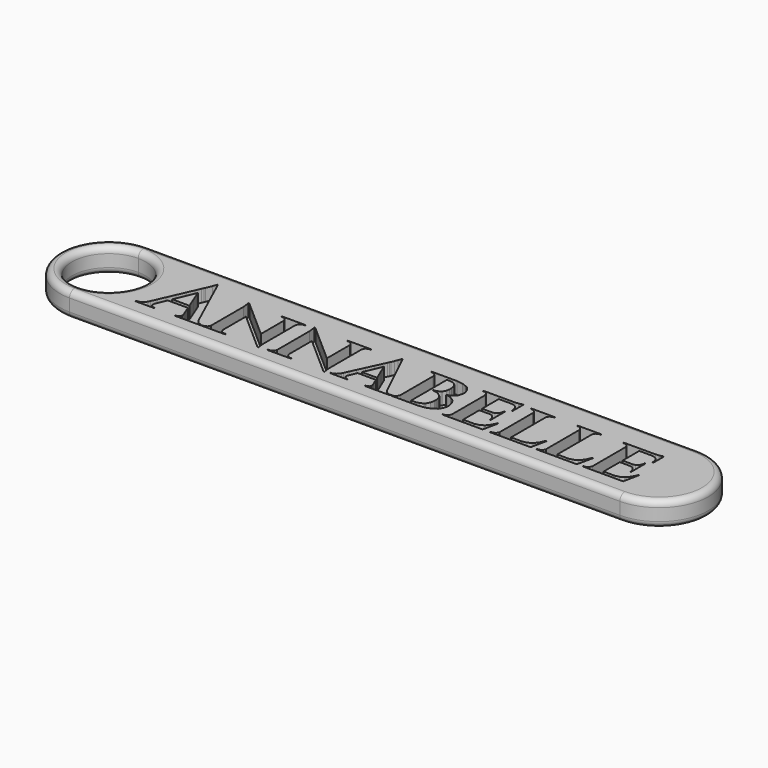
from build123d import *

# Parameters (mm, degrees)
F1_DEPTH = 6
F2_DEPTH = 3
F3_R     = 1.49999


# Not quite as in the source:
# - a fillet or chamfer is up to 0.001 mm smaller than in the source, because OpenCascade refuses the exact size


with BuildPart() as f1:
    # F0 (on Top) → F1 (new body)
    with BuildSketch(Plane.XY):
        with BuildLine():
            Line((62.0845109224, 12), (-72.4824666977, 12))
            Line((-72.4824666977, 12), (-72.4824666977, 9))
            ThreePointArc((-72.4824666977, 9), (-66.118505667, 6.3639610307), (-63.4824666977, 0))
            ThreePointArc((-63.4824666977, 0), (-66.118505667, -6.3639610307), (-72.4824666977, -9))
            Line((-72.4824666977, -9), (-72.4824666977, -12))
            Line((-72.4824666977, -12), (62.0845109224, -12))
            Line((62.0845109224, -12), (62.0845109224, 12))
        make_face()
        Polygon((-18.2442957235, 5.0671484936), (-18.2442957235, 5.1719728767), (-17.3239731739, 5.1719728767), (-15.297442463, 5.1719728767), (-13.2704675811, 5.1719728767), (-12.3490346036, 5.1719728767), (-12.3490346036, 5.0671484936), (-12.3490346036, 4.9623241106), (-12.5271472206, 4.9623241106), (-12.7054819232, 4.9623241106), (-12.9082460371, 4.9623241106), (-13.4587961337, 4.7178079119), (-13.5129850097, 4.6682828326), (-13.5669518002, 4.6200902667), (-13.8563292814, 3.9900335405), (-13.8601047359, 3.9129698521), (-13.8601047359, 3.5201005011), (-13.8601047359, 2.4802959216), (-13.8601047359, 1.0127101415), (-13.8601047359, -0.6717199768), (-13.8601047359, -2.3549286245), (-13.8601047359, -3.822492196), (-13.8601047359, -4.8623189841), (-13.8601047359, -5.2563431799), (-13.8601047359, -5.5527163562), (-13.8176863944, -6.4419247193), (-13.7199687492, -7.2564235009), (-13.6913197123, -7.3962263592), (-13.6706657554, -7.5432025811), (-13.6491234564, -7.6902010115), (-13.8381182657, -7.6902010115), (-14.2527520013, -7.3239153018), (-15.3443025156, -6.3611966192), (-16.8864646259, -5.0008781633), (-18.6540435768, -3.440571663), (-20.4229550411, -1.8802207456), (-21.9651171514, -0.5199022898), (-23.0568897513, 0.4428163928), (-23.4701909735, 0.8079028405), (-23.4701909735, 0.5102637766), (-23.4701909735, -0.2764965189), (-23.4701909735, -1.3886121559), (-23.4701909735, -2.6646047256), (-23.4701909735, -3.9393758248), (-23.4701909735, -5.0514914618), (-23.4701909735, -5.8382961744), (-23.4701909735, -6.1370900833), (-23.4664155191, -6.2141981888), (-23.1774822089, -6.8528274175), (-23.1230712474, -6.9033962989), (-23.0688823714, -6.954031806), (-22.5050071413, -7.2070538815), (-22.316012332, -7.2070538815), (-22.1372334583, -7.2070538815), (-21.9591208413, -7.2070538815), (-21.9591208413, -7.311856056), (-21.9591208413, -7.4179019096), (-22.8772225354, -7.4179019096), (-24.8966465084, -7.4179019096), (-26.9174029947, -7.4179019096), (-27.8341721755, -7.4179019096), (-27.8341721755, -7.311856056), (-27.8341721755, -7.2070538815), (-27.6667196652, -7.2070538815), (-27.4979346416, -7.2070538815), (-27.2942821855, -7.2070538815), (-26.736625351, -6.954031806), (-26.6799935339, -6.9033962989), (-26.6244721446, -6.8528274175), (-26.343756, -6.3154247858), (-26.343756, -6.1370900833), (-26.343756, -5.7394903099), (-26.343756, -4.6936450033), (-26.343756, -3.2152436565), (-26.343756, -1.5211528165), (-26.343756, 0.174115077), (-26.343756, 1.6525386322), (-26.343756, 2.6983839389), (-26.343756, 3.0948066588), (-26.343756, 3.6140426919), (-26.4834478157, 5.03583443), (-26.5112085103, 5.1719728767), (-26.5327508094, 5.3189935157), (-26.5534047662, 5.4660141546), (-26.4594625755, 5.4564644757), (-26.3652982992, 5.4455822833), (-25.9535516758, 5.0829165682), (-24.8639999315, 4.1250615593), (-23.3253911901, 2.7707838306), (-21.5602551803, 1.2175618596), (-19.7964516838, -0.33552686), (-18.257620857, -1.6898490059), (-17.1685132837, -2.6477262233), (-16.7552120615, -3.011613409), (-16.7552120615, -2.7139965536), (-16.7552120615, -1.9320110976), (-16.7552120615, -0.8259361878), (-16.7552120615, 0.4404178688), (-16.7552120615, 1.7079711874), (-16.7552120615, 2.8140905143), (-16.7552120615, 3.5960537617), (-16.7552120615, 3.8923158952), (-16.7552120615, 4.0839757312), (-17.026378527, 4.6080976466), (-17.080567403, 4.6587331537), (-17.134756279, 4.7093686607), (-17.6999640224, 4.9623241106), (-17.887848404, 4.9623241106), (-18.0661831065, 4.9623241106), (-18.2442957235, 4.9623241106), align=None, mode=Mode.SUBTRACT)
        Polygon((1.836236201, -7.2070538815), (2.0458849671, -7.2070538815), (2.2133374774, -7.2070538815), (2.2133374774, -7.311856056), (2.2133374774, -7.4179019096), (1.2494861585, -7.4179019096), (-0.8712088287, -7.4179019096), (-2.9916817302, -7.4179019096), (-3.9555330491, -7.4179019096), (-3.9555330491, -7.311856056), (-3.9555330491, -7.2070538815), (-3.7869701111, -7.2070538815), (-3.6350635899, -7.2070538815), (-3.2111022609, -6.9973829068), (-3.1786777695, -6.95643033), (-3.1471416204, -6.9142562827), (-2.9905713024, -6.5985616629), (-2.9905713024, -6.4937594884), (-2.9905713024, -6.3828943781), (-3.060528253, -6.0913182499), (-3.0738533865, -6.0539634592), (-3.2026630097, -5.7515273472), (-3.4833791542, -5.0876469906), (-3.7640952987, -4.423766634), (-3.8917944942, -4.122529784), (-4.0832322446, -4.122529784), (-4.588254802, -4.122529784), (-5.3004831845, -4.122529784), (-6.1173138644, -4.122529784), (-6.9341445443, -4.122529784), (-7.6461508412, -4.122529784), (-8.1511733986, -4.122529784), (-8.3415007213, -4.122529784), (-8.4729753712, -4.42736442), (-8.7607982535, -5.0985069743), (-9.0499536492, -5.768383641), (-9.1800957858, -6.0744397475), (-9.1947534326, -6.1093960143), (-9.2644882976, -6.4057691906), (-9.2644882976, -6.504575055), (-9.2644882976, -6.6190379513), (-9.0981462151, -6.9250940579), (-9.064611296, -6.9660466346), (-9.0317426335, -7.005822158), (-8.5931236577, -7.2070538815), (-8.4463251043, -7.2070538815), (-8.2777621663, -7.2070538815), (-8.2777621663, -7.311856056), (-8.2777621663, -7.4179019096), (-8.4583177244, -7.4179019096), (-8.9342470738, -7.4179019096), (-9.6065000559, -7.4179019096), (-10.3766927688, -7.4179019096), (-11.1466633961, -7.4179019096), (-11.8186942927, -7.4179019096), (-12.2946236421, -7.4179019096), (-12.4740687724, -7.4179019096), (-12.4740687724, -7.311856056), (-12.4740687724, -7.2070538815), (-12.3066162622, -7.2070538815), (-12.0874178171, -7.2070538815), (-11.4995573468, -6.9793051424), (-11.4260470273, -6.9347547796), (-11.3525367078, -6.8889385291), (-10.7573474141, -6.2069804082), (-10.7113757037, -6.1166137949), (-10.5259342634, -5.715394027), (-10.0331264116, -4.6599102071), (-9.3377765315, -3.1682281441), (-8.5400452095, -1.4585246893), (-7.7425359731, 0.252444653), (-7.0476302641, 1.744082299), (-6.5546003268, 2.7996549531), (-6.3678263731, 3.1996310419), (-6.2643345034, 3.4332650482), (-5.962964402, 4.1394971206), (-5.6667022685, 4.8792641121), (-5.4799283148, 5.4202645298), (-5.4099713642, 5.680548803), (-5.4028646264, 5.7600554326), (-5.2147581593, 5.7600554326), (-4.9737953296, 5.2539224474), (-4.3366318656, 3.9176336488), (-3.4365191016, 2.0296399086), (-2.4038212599, -0.1355388157), (-1.3711234182, -2.3007175399), (-0.4710106543, -4.1887779057), (0.1661528097, -5.5250222872), (0.4084481528, -6.0322657002), (0.4530873498, -6.1334700887), (1.0567158947, -6.8769014919), (1.1326691553, -6.9238947959), (1.2072899026, -6.9708880998), align=None, mode=Mode.SUBTRACT)
        Polygon((12.7053254633, 2.3874641586), (12.7053254633, 2.045319149), (12.7053254633, 1.7043289842), (12.4248314044, 0.7801643544), (12.3695321006, 0.6813806985), (12.260932263, 0.4934296913), (11.550036394, -0.1933698948), (10.6161666253, -0.5379800541), (10.3969681802, -0.5560356099), (10.6308242721, -0.5729141123), (11.687507354, -0.8572724599), (12.5887305457, -1.4030921342), (12.7464112914, -1.5525112972), (12.9032036949, -1.7006867811), (13.4548642194, -2.5681973852), (13.6911632524, -3.5140375654), (13.6911632524, -3.8297321852), (13.6911632524, -4.1357882918), (13.4877328818, -5.0563107184), (12.8778859414, -6.0322657002), (11.8609561743, -6.7564200771), (10.8031626646, -7.1504220643), (10.4391644361, -7.2287294319), (10.2850370593, -7.260065704), (8.8894514169, -7.4179019096), (8.4246263454, -7.4179019096), (7.4727676466, -7.4179019096), (5.3820542097, -7.4179019096), (3.2904524305, -7.4179019096), (2.3399262451, -7.4179019096), (2.3399262451, -7.311856056), (2.3399262451, -7.2070538815), (2.4543003071, -7.2070538815), (2.5700068825, -7.2070538815), (2.7709943119, -7.2070538815), (3.3242094353, -6.9443710842), (3.3783983113, -6.8925807323), (3.4328092728, -6.8395467012), (3.7208542407, -6.175644136), (3.724185524, -6.0961152979), (3.724185524, -5.668400723), (3.724185524, -4.5418273163), (3.724185524, -2.9489630733), (3.724185524, -1.1223315726), (3.724185524, 0.7042555109), (3.724185524, 2.2970753368), (3.724185524, 3.4237153692), (3.724185524, 3.8503417249), (3.7208542407, 3.976708407), (3.5351907147, 4.4852843334), (3.1254428614, 4.8335144873), (3.0110687994, 4.8779315988), (2.9762013669, 4.8925892455), (2.6710558111, 4.9623241106), (2.5700068825, 4.9623241106), (2.4543003071, 4.9623241106), (2.3399262451, 4.9623241106), (2.3399262451, 5.0671484936), (2.3399262451, 5.1719728767), (3.2182746244, 5.1719728767), (5.1508631445, 5.1719728767), (7.0834516645, 5.1719728767), (7.9629104716, 5.1719728767), (8.4812581625, 5.1719728767), (10.037855834, 4.9767596718), (11.5200548437, 4.3913421426), (12.4092854154, 3.4141656903), align=None, mode=Mode.SUBTRACT)
        Polygon((24.8882728829, -7.2516264528), (24.8545158782, -7.4179019096), (24.4289999503, -7.4179019096), (23.3096887412, -7.4179019096), (21.7266628884, -7.4179019096), (19.9120017993, -7.4179019096), (18.0975627958, -7.4179019096), (16.5140927719, -7.4179019096), (15.3947815628, -7.4179019096), (14.9705981483, -7.4179019096), (14.9705981483, -7.311856056), (14.9705981483, -7.2070538815), (15.0958544026, -7.2070538815), (15.2226652559, -7.2070538815), (15.4238747708, -7.2070538815), (15.9768678086, -6.9443710842), (16.0310566846, -6.8925807323), (16.0854676462, -6.8395467012), (16.3732905285, -6.1925226384), (16.3768438974, -6.1166137949), (16.3768438974, -5.6864784874), (16.3768438974, -4.5550636155), (16.3768438974, -2.9549593833), (16.3768438974, -1.1223315726), (16.3768438974, 0.7115177086), (16.3768438974, 2.311510898), (16.3768438974, 3.4430368127), (16.3768438974, 3.871884024), (16.3732905285, 3.9489477124), (16.0854676462, 4.5961050265), (16.0310566846, 4.6478509613), (15.9768678086, 4.7009294096), (15.4105496374, 4.9623241106), (15.2226652559, 4.9623241106), (15.0958544026, 4.9623241106), (14.9705981483, 4.9623241106), (14.9705981483, 5.0671484936), (14.9705981483, 5.1719728767), (15.2877363242, 5.1719728767), (16.1238884476, 5.1719728767), (17.3069382116, 5.1719728767), (18.663880967, 5.1719728767), (20.019047038, 5.1719728767), (21.2023188875, 5.1719728767), (22.038471011, 5.1719728767), (22.3569417002, 5.1719728767), (22.6663068816, 5.1719728767), (23.4833596471, 5.2599187574), (23.595290768, 5.2767972598), (23.7063335467, 5.2950082755), (24.4929605908, 5.4695675235), (24.5389323012, 5.4864460259), (24.5389323012, 5.3443112692), (24.5389323012, 4.966099565), (24.5389323012, 4.4322058852), (24.5389323012, 3.8190276613), (24.5389323012, 3.2067377797), (24.5389323012, 2.6730661854), (24.5389323012, 2.2946323957), (24.5389323012, 2.1513872112), (24.4341079181, 2.1513872112), (24.3290614495, 2.1513872112), (24.3290614495, 2.3392715927), (24.3290614495, 2.5453669899), (24.2026947673, 3.163431096), (23.9086534894, 3.7008781448), (23.8253714054, 3.7874915122), (23.7412009792, 3.8756594784), (23.2217428605, 4.1863571732), (22.5699217497, 4.3298244432), (22.4206802552, 4.3322673843), (21.9480821891, 4.3322673843), (20.9096101229, 4.3322673843), (19.8698055434, 4.3322673843), (19.3987620763, 4.3322673843), (19.3987620763, 3.5358685757), (19.3987620763, 1.7838356138), (19.3987620763, 0.0319581117), (19.3987620763, -0.7657065846), (19.7723099838, -0.7657065846), (20.5940265459, -0.7657065846), (21.4157431081, -0.7657065846), (21.790623529, -0.7657065846), (21.9083288743, -0.76208659), (22.4348937308, -0.634365186), (22.871291851, -0.3596453516), (22.9448021705, -0.2837365081), (23.01831249, -0.2066284026), (23.2748213087, 0.2415846693), (23.3856420018, 0.7295732645), (23.3856420018, 0.8922287267), (23.3856420018, 1.0380278951), (23.4904663849, 1.0380278951), (23.595290768, 1.0380278951), (23.595290768, 0.8476561553), (23.595290768, 0.3440105283), (23.595290768, -0.3680846028), (23.595290768, -1.1850041169), (23.595290768, -2.0019236311), (23.595290768, -2.7139965536), (23.595290768, -3.2176421806), (23.595290768, -3.4092353909), (23.4904663849, -3.4092353909), (23.3856420018, -3.4092353909), (23.3856420018, -3.2634140139), (23.3856420018, -3.0501674618), (23.2013109892, -2.4127819122), (22.772463778, -1.9091362852), (22.6507608926, -1.8356259657), (22.5870223376, -1.797071913), (22.0049360918, -1.6055009112), (21.812165828, -1.6055009112), (21.4348424661, -1.6055009112), (20.6049087383, -1.6055009112), (19.7745308393, -1.6055009112), (19.3987620763, -1.6055009112), (19.3987620763, -2.3814678486), (19.3987620763, -4.0911935118), (19.3987620763, -5.8009413837), (19.3987620763, -6.5780853745), (19.7914093417, -6.5780853745), (20.6579871865, -6.5780853745), (21.5227883468, -6.5780853745), (21.9169902111, -6.5780853745), (22.1326352873, -6.5744653799), (23.1193614186, -6.3648166138), (23.9772779266, -5.9009243016), (24.1305169612, -5.7708043735), (24.2822013969, -5.6394851835), (24.9195869465, -4.8225656693), (25.3917408414, -3.793598865), (25.4630303053, -3.5562338213), (25.6509146868, -3.5562338213), (25.6160472543, -3.7212878075), (25.5256584325, -4.1586631042), (25.397959237, -4.777993098), (25.2520490258, -5.4864682345), (25.1063609002, -6.1949211624), (24.9786617047, -6.8142511562), align=None, mode=Mode.SUBTRACT)
        Polygon((27.1246744454, -7.4179019096), (26.7004910309, -7.4179019096), (26.7004910309, -7.311856056), (26.7004910309, -7.2070538815), (26.8257472852, -7.2070538815), (26.9521139673, -7.2070538815), (27.1533234823, -7.2070538815), (27.7052060923, -6.9443710842), (27.7593949683, -6.8925807323), (27.8138059299, -6.8395467012), (28.0860828232, -6.29736923), (28.0860828232, -6.1166137949), (28.0860828232, -5.6876777494), (28.0860828232, -4.5587058186), (28.0860828232, -2.9622215811), (28.0860828232, -1.1331915564), (28.0860828232, 0.6970377303), (28.0860828232, 2.2935219679), (28.0860828232, 3.4223828559), (28.0860828232, 3.8503417249), (28.0860828232, 4.0477757854), (27.8053666787, 4.582779893), (27.7498452893, 4.636968769), (27.6932134722, 4.691157645), (27.1366670655, 4.9623241106), (26.9521139673, 4.9623241106), (26.8257472852, 4.9623241106), (26.7004910309, 4.9623241106), (26.7004910309, 5.0671484936), (26.7004910309, 5.1719728767), (27.6112639016, 5.1719728767), (29.6162523133, 5.1719728767), (31.6212407251, 5.1719728767), (32.5333461091, 5.1719728767), (32.5333461091, 5.0671484936), (32.5333461091, 4.9623241106), (32.4067573414, 4.9623241106), (32.2812790015, 4.9623241106), (32.0765161176, 4.9623241106), (31.5188592831, 4.7009294096), (31.4633378938, 4.6478509613), (31.4064839911, 4.5961050265), (31.1284328733, 4.0368935931), (31.1284328733, 3.8503417249), (31.1284328733, 3.403283498), (31.1284328733, 2.2211220762), (31.1284328733, 0.5512607705), (31.1284328733, -1.3633166109), (31.1284328733, -3.2778939923), (31.1284328733, -4.9478885493), (31.1284328733, -6.1298723027), (31.1284328733, -6.5780853745), (31.5210801387, -6.5780853745), (32.3861033846, -6.5780853745), (33.251348716, -6.5780853745), (33.6453284948, -6.5780853745), (33.8620839987, -6.5744653799), (34.84681136, -6.3648166138), (35.6982873869, -5.9009243016), (35.8490834804, -5.7708043735), (35.9985470605, -5.6394851835), (36.6299363, -4.8225656693), (37.1009797671, -3.793598865), (37.1709367177, -3.5562338213), (37.2866432931, -3.5562338213), (37.4023498685, -3.5562338213), (37.3661499226, -3.7212878075), (37.2733181596, -4.1586631042), (37.1418435097, -4.777993098), (36.9926020152, -5.4864682345), (36.8418059217, -6.1949211624), (36.7107754429, -6.8142511562), (36.6179436799, -7.2516264528), (36.5830762474, -7.4179019096), (36.1575603195, -7.4179019096), (35.0382491105, -7.4179019096), (33.4550011721, -7.4179019096), (31.6416725964, -7.4179019096), (29.8270115072, -7.4179019096), (28.2437635689, -7.4179019096), align=None, mode=Mode.SUBTRACT)
        Polygon((38.4350477101, -7.4179019096), (38.0108642956, -7.4179019096), (38.0108642956, -7.311856056), (38.0108642956, -7.2070538815), (38.13612055, -7.2070538815), (38.2624872321, -7.2070538815), (38.463696747, -7.2070538815), (39.0153572715, -6.9443710842), (39.0697682331, -6.8925807323), (39.123957109, -6.8395467012), (39.3951235746, -6.29736923), (39.3951235746, -6.1166137949), (39.3951235746, -5.6876777494), (39.3951235746, -4.5587058186), (39.3951235746, -2.9622215811), (39.3951235746, -1.1331915564), (39.3951235746, 0.6970377303), (39.3951235746, 2.2935219679), (39.3951235746, 3.4223828559), (39.3951235746, 3.8503417249), (39.3951235746, 4.0477757854), (39.1144074301, 4.582779893), (39.0588860407, 4.636968769), (39.0022542236, 4.691157645), (38.4470403302, 4.9623241106), (38.2624872321, 4.9623241106), (38.13612055, 4.9623241106), (38.0108642956, 4.9623241106), (38.0108642956, 5.0671484936), (38.0108642956, 5.1719728767), (38.9216371663, 5.1719728767), (40.9266255781, 5.1719728767), (42.9316139898, 5.1719728767), (43.8437193739, 5.1719728767), (43.8437193739, 5.0671484936), (43.8437193739, 4.9623241106), (43.7171306062, 4.9623241106), (43.5916522663, 4.9623241106), (43.3868893824, 4.9623241106), (42.8292325479, 4.7009294096), (42.7737111585, 4.6478509613), (42.7168572559, 4.5961050265), (42.4374736247, 4.0368935931), (42.4374736247, 3.8503417249), (42.4374736247, 3.403283498), (42.4374736247, 2.2211220762), (42.4374736247, 0.5512607705), (42.4374736247, -1.3633166109), (42.4374736247, -3.2778939923), (42.4374736247, -4.9478885493), (42.4374736247, -6.1298723027), (42.4374736247, -6.5780853745), (42.8303429757, -6.5780853745), (43.6964766493, -6.5780853745), (44.5617219808, -6.5780853745), (44.9557017595, -6.5780853745), (45.1724572635, -6.5744653799), (46.1569625392, -6.3648166138), (47.0086606517, -5.9009243016), (47.1594567451, -5.7708043735), (47.3089203252, -5.6394851835), (47.9403095648, -4.8225656693), (48.4100205185, -3.793598865), (48.4813099825, -3.5562338213), (48.5956840445, -3.5562338213), (48.7113906199, -3.5562338213), (48.675190674, -3.7212878075), (48.5823589111, -4.1586631042), (48.4522167744, -4.777993098), (48.3016427666, -5.4864682345), (48.1512908442, -6.1949211624), (48.0209266221, -6.8142511562), (47.9280948591, -7.2516264528), (47.8932274266, -7.4179019096), (47.4679335843, -7.4179019096), (46.3486223752, -7.4179019096), (44.7653744369, -7.4179019096), (42.9518237755, -7.4179019096), (41.137384772, -7.4179019096), (39.5539147481, -7.4179019096), align=None, mode=Mode.SUBTRACT)
        Polygon((59.2373576961, -7.2516264528), (59.2036006913, -7.4179019096), (58.778306849, -7.4179019096), (57.65899564, -7.4179019096), (56.0757477016, -7.4179019096), (54.2610866125, -7.4179019096), (52.4464255234, -7.4179019096), (50.8633996706, -7.4179019096), (49.7440884616, -7.4179019096), (49.319905047, -7.4179019096), (49.319905047, -7.311856056), (49.319905047, -7.2070538815), (49.4451613014, -7.2070538815), (49.5715279835, -7.2070538815), (49.7727374985, -7.2070538815), (50.3257305363, -6.9443710842), (50.3801414978, -6.8925807323), (50.4343303738, -6.8395467012), (50.7221532561, -6.1925226384), (50.7259287106, -6.1166137949), (50.7259287106, -5.6864784874), (50.7259287106, -4.5550636155), (50.7259287106, -2.9549593833), (50.7259287106, -1.1223315726), (50.7259287106, 0.7115177086), (50.7259287106, 2.311510898), (50.7259287106, 3.4430368127), (50.7259287106, 3.871884024), (50.7221532561, 3.9489477124), (50.4343303738, 4.5961050265), (50.3801414978, 4.6478509613), (50.3257305363, 4.7009294096), (49.759412365, 4.9623241106), (49.5715279835, 4.9623241106), (49.4451613014, 4.9623241106), (49.319905047, 4.9623241106), (49.319905047, 5.0671484936), (49.319905047, 5.1719728767), (49.6365990518, 5.1719728767), (50.4729732608, 5.1719728767), (51.6560230248, 5.1719728767), (53.0127436946, 5.1719728767), (54.3683539367, 5.1719728767), (55.5516257863, 5.1719728767), (56.3877779097, 5.1719728767), (56.7058044278, 5.1719728767), (57.0153916948, 5.1719728767), (57.8322223747, 5.2599187574), (57.9445976667, 5.2767972598), (58.0551962743, 5.2950082755), (58.842045404, 5.4695675235), (58.8877950288, 5.4864460259), (58.8877950288, 5.3443112692), (58.8877950288, 4.966099565), (58.8877950288, 4.4322058852), (58.8877950288, 3.8190276613), (58.8877950288, 3.2067377797), (58.8877950288, 2.6730661854), (58.8877950288, 2.2946323957), (58.8877950288, 2.1513872112), (58.7829706457, 2.1513872112), (58.6781462626, 2.1513872112), (58.6781462626, 2.3392715927), (58.6781462626, 2.5453669899), (58.551557495, 3.163431096), (58.2577383026, 3.7008781448), (58.1746783041, 3.7874915122), (58.0900637068, 3.8756594784), (57.5710497593, 4.1863571732), (56.9190065629, 4.3298244432), (56.7697650683, 4.3322673843), (56.2973890879, 4.3322673843), (55.2589170217, 4.3322673843), (54.2186682711, 4.3322673843), (53.7478468895, 4.3322673843), (53.7478468895, 3.5358685757), (53.7478468895, 1.7838356138), (53.7478468895, 0.0319581117), (53.7478468895, -0.7657065846), (54.1213947969, -0.7657065846), (54.9431113591, -0.7657065846), (55.7648279213, -0.7657065846), (56.1394862566, -0.7657065846), (56.2576357731, -0.76208659), (56.7842006296, -0.634365186), (57.2203766642, -0.3596453516), (57.2936648981, -0.2837365081), (57.3671752176, -0.2066284026), (57.6236840363, 0.2415846693), (57.734726815, 0.7295732645), (57.734726815, 0.8922287267), (57.734726815, 1.0380278951), (57.8397732837, 1.0380278951), (57.9445976667, 1.0380278951), (57.9445976667, 0.8476561553), (57.9445976667, 0.3440105283), (57.9445976667, -0.3680846028), (57.9445976667, -1.1850041169), (57.9445976667, -2.0019236311), (57.9445976667, -2.7139965536), (57.9445976667, -3.2176421806), (57.9445976667, -3.4092353909), (57.8397732837, -3.4092353909), (57.734726815, -3.4092353909), (57.734726815, -3.2634140139), (57.734726815, -3.0501674618), (57.5503958024, -2.4127819122), (57.1215485912, -1.9091362852), (56.9998457058, -1.8356259657), (56.9358850652, -1.797071913), (56.3537988194, -1.6055009112), (56.1599181279, -1.6055009112), (55.7828168515, -1.6055009112), (54.9537714659, -1.6055009112), (54.1238377381, -1.6055009112), (53.7478468895, -1.6055009112), (53.7478468895, -2.3814678486), (53.7478468895, -4.0911935118), (53.7478468895, -5.8009413837), (53.7478468895, -6.5780853745), (54.1407162404, -6.5780853745), (55.0055174007, -6.5780853745), (55.8707627322, -6.5780853745), (56.2647425109, -6.5780853745), (56.4814980149, -6.5744653799), (57.4686683173, -6.3648166138), (58.3263627398, -5.9009243016), (58.4793796888, -5.7708043735), (58.6310641245, -5.6394851835), (59.2675613319, -4.8225656693), (59.7410477401, -3.793598865), (59.8107826051, -3.5562338213), (59.9999995, -3.5562338213), (59.9649099819, -3.7212878075), (59.8745211601, -4.1586631042), (59.7468219646, -4.777993098), (59.601133839, -5.4864682345), (59.4554457134, -6.1949211624), (59.3277465179, -6.8142511562), align=None, mode=Mode.SUBTRACT)
        Polygon((-43.9700204303, -7.2070538815), (-43.9484781313, -7.2070538815), (-43.8025679201, -7.2070538815), (-43.7592612364, -7.2070538815), (-43.6340049821, -7.2070538815), (-43.430352526, -7.2070538815), (-42.8724736059, -6.954031806), (-42.8158417888, -6.9033962989), (-42.7603203994, -6.8528274175), (-42.4796042549, -6.3154247858), (-42.4796042549, -6.1370900833), (-42.4796042549, -5.7394903099), (-42.4796042549, -4.6936450033), (-42.4796042549, -3.2152436565), (-42.4796042549, -1.5211528165), (-42.4796042549, 0.174115077), (-42.4796042549, 1.6525386322), (-42.4796042549, 2.6983839389), (-42.4796042549, 3.0948066588), (-42.4796042549, 3.6140426919), (-42.6206285839, 5.03583443), (-42.6483892785, 5.1719728767), (-42.6688211498, 5.3189935157), (-42.6892530211, 5.4660141546), (-42.5953108303, 5.4564644757), (-42.5002582118, 5.4455822833), (-42.0880674173, 5.0829165682), (-40.9989598441, 4.1250615593), (-39.4601290172, 2.7707838306), (-37.6963255207, 1.2175618596), (-35.9322999387, -0.33552686), (-34.3936911974, -1.6898490059), (-33.3045836241, -2.6477262233), (-32.8912824019, -3.011613409), (-32.8912824019, -2.7139965536), (-32.8912824019, -1.9320110976), (-32.8912824019, -0.8259361878), (-32.8912824019, 0.4404178688), (-32.8912824019, 1.7079711874), (-32.8912824019, 2.8140905143), (-32.8912824019, 3.5960537617), (-32.8912824019, 3.8923158952), (-32.8912824019, 4.0839757312), (-33.1624488674, 4.6080976466), (-33.2164156579, 4.6587331537), (-33.2706045339, 4.7093686607), (-33.8355901918, 4.9623241106), (-34.0239187444, 4.9623241106), (-34.2022534469, 4.9623241106), (-34.3803660639, 4.9623241106), (-34.3803660639, 5.0671484936), (-34.3803660639, 5.1719728767), (-33.4595993432, 5.1719728767), (-31.4330686323, 5.1719728767), (-29.4065379215, 5.1719728767), (-28.4848828585, 5.1719728767), (-28.4848828585, 5.0671484936), (-28.4848828585, 4.9623241106), (-28.6632175611, 4.9623241106), (-28.8415522636, 4.9623241106), (-29.0438722064, 4.9623241106), (-29.594422303, 4.7178079119), (-29.6488332646, 4.6682828326), (-29.7030221406, 4.6200902667), (-29.9921775362, 3.9900335405), (-29.9946204774, 3.9129698521), (-29.9946204774, 3.5201005011), (-29.9946204774, 2.4802959216), (-29.9946204774, 1.0127101415), (-29.9946204774, -0.6717199768), (-29.9946204774, -2.3549286245), (-29.9946204774, -3.822492196), (-29.9946204774, -4.8623189841), (-29.9946204774, -5.2563431799), (-29.9946204774, -5.5527163562), (-29.9535346493, -6.4419247193), (-29.8560390896, -7.2564235009), (-29.8271679671, -7.3962263592), (-29.8067360959, -7.5432025811), (-29.7847496257, -7.6902010115), (-29.9741886061, -7.6902010115), (-30.3883781706, -7.3239153018), (-31.4790403427, -6.3611966192), (-33.0225349663, -5.0008781633), (-34.7901139172, -3.440571663), (-36.5574707826, -1.8802207456), (-38.1011874918, -0.5199022898), (-39.1914054928, 0.4428163928), (-39.604706715, 0.8079028405), (-39.604706715, 0.5102637766), (-39.604706715, -0.2764965189), (-39.604706715, -1.3886121559), (-39.604706715, -2.6646047256), (-39.604706715, -3.9393758248), (-39.604706715, -5.0514914618), (-39.604706715, -5.8382961744), (-39.604706715, -6.1370900833), (-39.6024858595, -6.2141981888), (-39.3133304638, -6.8528274175), (-39.2589195023, -6.9033962989), (-39.2047306263, -6.954031806), (-38.6397449684, -7.2070538815), (-38.4505280735, -7.2070538815), (-38.2733037987, -7.2070538815), (-38.0949690962, -7.2070538815), (-38.0949690962, -7.311856056), (-38.0949690962, -7.4179019096), (-39.0132928758, -7.4179019096), (-41.0324947633, -7.4179019096), (-43.0532512496, -7.4179019096), (-43.7592612364, -7.4179019096), (-43.9700204303, -7.4179019096), (-44.0473062043, -7.4179019096), (-44.8063946393, -7.4179019096), (-45.8775132824, -7.4179019096), (-47.1064459226, -7.4179019096), (-48.3366444504, -7.4179019096), (-49.4077853021, -7.4179019096), (-50.1668959456, -7.4179019096), (-50.4536306087, -7.4179019096), (-50.4536306087, -7.311856056), (-50.4536306087, -7.2070538815), (-50.2644803395, -7.2070538815), (-50.0945848882, -7.2070538815), (-49.6198548008, -6.9708880998), (-49.58250001, -6.9238947959), (-49.5463444813, -6.8769014919), (-49.3620134687, -6.5106157822), (-49.3620134687, -6.3889128967), (-49.3620134687, -6.2624129633), (-49.4499593494, -5.9274635257), (-49.4668156432, -5.8852672698), (-49.5114326317, -5.7732251061), (-49.6282940519, -5.4816267693), (-49.7921487762, -5.0683699642), (-49.9813212539, -4.5948169302), (-50.1704937317, -4.1201090514), (-50.3343484559, -3.7068300377), (-50.4512098762, -3.4152317009), (-50.4946276026, -3.3043887993), (-50.7066748928, -3.3043887993), (-51.2621108717, -3.3043887993), (-52.0489155843, -3.3043887993), (-52.9501831931, -3.3043887993), (-53.852650064, -3.3043887993), (-54.639432568, -3.3043887993), (-55.1948685469, -3.3043887993), (-55.4057387836, -3.3043887993), (-55.4527320876, -3.4152317009), (-55.576833497, -3.7068300377), (-55.7515259964, -4.1201090514), (-55.9515584579, -4.5948169302), (-56.1515687109, -5.0683699642), (-56.3262834189, -5.4816267693), (-56.4503848283, -5.7732251061), (-56.4961788702, -5.8852672698), (-56.514234426, -5.9298620497), (-56.6009810447, -6.2816899897), (-56.6009810447, -6.3997728805), (-56.6009810447, -6.5298928086), (-56.409410043, -6.8769014919), (-56.3708559902, -6.9238947959), (-56.3322797289, -6.9708880998), (-55.8419148183, -7.2070538815), (-55.6780378855, -7.2070538815), (-55.5105631667, -7.2070538815), (-55.5105631667, -7.311856056), (-55.5105631667, -7.4179019096), (-55.7045549011, -7.4179019096), (-56.2130197846, -7.4179019096), (-56.9311112258, -7.4179019096), (-57.7552707291, -7.4179019096), (-58.5806294944, -7.4179019096), (-59.2987431441, -7.4179019096), (-59.8072080277, -7.4179019096), (-60.0000005, -7.4179019096), (-60.0000005, -7.311856056), (-60.0000005, -7.2070538815), (-59.8120272843, -7.2070538815), (-59.571042246, -7.2070538815), (-58.9276381778, -6.9624488486), (-58.8469100777, -6.9142562827), (-58.7674034481, -6.8648422462), (-58.1022794124, -6.1298723027), (-58.0492675899, -6.0322657002), (-57.8420395563, -5.5599341368), (-57.2925998875, -4.3164993098), (-56.5166551586, -2.5597803426), (-55.6262475335, -0.5451978347), (-54.7358399085, 1.4705839351), (-53.9598507625, 3.2273917365), (-53.4104555107, 4.4708487721), (-53.2019837981, 4.9418922393), (-53.0381512824, 5.2887898799), (-52.4465375662, 6.6672749343), (-52.1633784806, 7.5782698906), (-52.1525407054, 7.6902010115), (-51.9645674896, 7.6902010115), (-51.6970876443, 7.103450969), (-50.9910110319, 5.5528496075), (-49.9933804997, 3.3621976698), (-48.84870712, 0.8500546793), (-47.7040781574, -1.6621327283), (-46.7064254167, -3.8526292061), (-46.0003265956, -5.4033194018), (-45.7316030712, -5.9913131234), (-45.6798571364, -6.0925175119), (-45.0160434054, -6.8528274175), (-44.9352042626, -6.9033962989), (-44.855697633, -6.954031806), (-44.1761158275, -7.2070538815), align=None, mode=Mode.SUBTRACT)
        with BuildLine():
            ThreePointArc((62.0845109224, -12), (74.0845109224, 0), (62.0845109224, 12))
            Line((62.0845109224, 12), (62.0845109224, -12))
        make_face()
        Polygon((12.7053254633, 1.7043289842), (12.7053254633, 2.045319149), (12.7053254633, 2.3874641586), (12.4092854154, 3.4141656903), (11.5200548437, 4.3913421426), (10.037855834, 4.9767596718), (8.4812581625, 5.1719728767), (7.9629104716, 5.1719728767), (7.0834516645, 5.1719728767), (5.1508631445, 5.1719728767), (3.2182746244, 5.1719728767), (2.3399262451, 5.1719728767), (2.3399262451, 5.0671484936), (2.3399262451, 4.9623241106), (2.4543003071, 4.9623241106), (2.5700068825, 4.9623241106), (2.6710558111, 4.9623241106), (2.9762013669, 4.8925892455), (3.0110687994, 4.8779315988), (3.1254428614, 4.8335144873), (3.5351907147, 4.4852843334), (3.7208542407, 3.976708407), (3.724185524, 3.8503417249), (3.724185524, 3.4237153692), (3.724185524, 2.2970753368), (3.724185524, 0.7042555109), (3.724185524, -1.1223315726), (3.724185524, -2.9489630733), (3.724185524, -4.5418273163), (3.724185524, -5.668400723), (3.724185524, -6.0961152979), (3.7208542407, -6.175644136), (3.4328092728, -6.8395467012), (3.3783983113, -6.8925807323), (3.3242094353, -6.9443710842), (2.7709943119, -7.2070538815), (2.5700068825, -7.2070538815), (2.4543003071, -7.2070538815), (2.3399262451, -7.2070538815), (2.3399262451, -7.311856056), (2.3399262451, -7.4179019096), (3.2904524305, -7.4179019096), (5.3820542097, -7.4179019096), (7.4727676466, -7.4179019096), (8.4246263454, -7.4179019096), (8.8894514169, -7.4179019096), (10.2850370593, -7.260065704), (10.4391644361, -7.2287294319), (10.8031626646, -7.1504220643), (11.8609561743, -6.7564200771), (12.8778859414, -6.0322657002), (13.4877328818, -5.0563107184), (13.6911632524, -4.1357882918), (13.6911632524, -3.8297321852), (13.6911632524, -3.5140375654), (13.4548642194, -2.5681973852), (12.9032036949, -1.7006867811), (12.7464112914, -1.5525112972), (12.5887305457, -1.4030921342), (11.687507354, -0.8572724599), (10.6308242721, -0.5729141123), (10.3969681802, -0.5560356099), (10.6161666253, -0.5379800541), (11.550036394, -0.1933698948), (12.260932263, 0.4934296913), (12.3695321006, 0.6813806985), (12.4248314044, 0.7801643544), align=None)
        Polygon((10.2921437971, -3.4188516955), (10.2921437971, -3.6405597074), (10.2921437971, -3.9682913644), (10.1004839611, -4.9514863354), (9.6536478197, -5.7455088285), (9.5259486243, -5.8647909814), (9.3982494288, -5.9828516637), (8.6462677316, -6.3997728805), (7.8185548594, -6.5780853745), (7.5425025116, -6.5780853745), (7.4110278616, -6.5780853745), (7.1234270649, -6.5780853745), (6.8340495836, -6.5780853745), (6.703907447, -6.5780853745), (6.703907447, -6.1081745437), (6.703907447, -4.8695589732), (6.703907447, -3.1188585247), (6.703907447, -1.111516006), (6.703907447, 0.8958487212), (6.703907447, 2.6466380041), (6.703907447, 3.8852091574), (6.703907447, 4.3538096834), (6.9981708105, 4.3538096834), (7.2919900029, 4.3538096834), (7.5413920838, 4.3538096834), (8.2920412676, 4.1972393655), (9.0064905056, 3.724863385), (9.4355598024, 2.9382363409), (9.5790270725, 2.1116338964), (9.5790270725, 1.8356703828), (9.5790270725, 1.566969067), (9.4211242412, 0.760887328), (9.0535726438, 0.1090662172), (8.9487482607, 0.0102381442), (8.8439238776, -0.0873462497), (8.2245272582, -0.4295134679), (7.5400595704, -0.5777333689), (7.3124218742, -0.5777333689), (7.3124218742, -0.7657065846), (7.3197506976, -0.7657065846), (7.3439580233, -0.7657065846), (7.3546181301, -0.7657065846), (7.7377157165, -0.7657065846), (8.8907839302, -1.0801575253), (9.7704648229, -1.8151496773), (9.8932781361, -2.0247984435), (9.9596817178, -2.1332650297), (10.1922052963, -2.7537720769), align=None, mode=Mode.SUBTRACT)
        with BuildLine():
            Line((-72.4824666977, 9), (-72.4824666977, 12))
            ThreePointArc((-72.4824666977, 12), (-84.4824666977, 0), (-72.4824666977, -12))
            Line((-72.4824666977, -12), (-72.4824666977, -9))
            ThreePointArc((-72.4824666977, -9), (-81.4824666977, 0), (-72.4824666977, 9))
        make_face()
        Polygon((-17.3239731739, 5.1719728767), (-18.2442957235, 5.1719728767), (-18.2442957235, 5.0671484936), (-18.2442957235, 4.9623241106), (-18.0661831065, 4.9623241106), (-17.887848404, 4.9623241106), (-17.6999640224, 4.9623241106), (-17.134756279, 4.7093686607), (-17.080567403, 4.6587331537), (-17.026378527, 4.6080976466), (-16.7552120615, 4.0839757312), (-16.7552120615, 3.8923158952), (-16.7552120615, 3.5960537617), (-16.7552120615, 2.8140905143), (-16.7552120615, 1.7079711874), (-16.7552120615, 0.4404178688), (-16.7552120615, -0.8259361878), (-16.7552120615, -1.9320110976), (-16.7552120615, -2.7139965536), (-16.7552120615, -3.011613409), (-17.1685132837, -2.6477262233), (-18.257620857, -1.6898490059), (-19.7964516838, -0.33552686), (-21.5602551803, 1.2175618596), (-23.3253911901, 2.7707838306), (-24.8639999315, 4.1250615593), (-25.9535516758, 5.0829165682), (-26.3652982992, 5.4455822833), (-26.4594625755, 5.4564644757), (-26.5534047662, 5.4660141546), (-26.5327508094, 5.3189935157), (-26.5112085103, 5.1719728767), (-26.4834478157, 5.03583443), (-26.343756, 3.6140426919), (-26.343756, 3.0948066588), (-26.343756, 2.6983839389), (-26.343756, 1.6525386322), (-26.343756, 0.174115077), (-26.343756, -1.5211528165), (-26.343756, -3.2152436565), (-26.343756, -4.6936450033), (-26.343756, -5.7394903099), (-26.343756, -6.1370900833), (-26.343756, -6.3154247858), (-26.6244721446, -6.8528274175), (-26.6799935339, -6.9033962989), (-26.736625351, -6.954031806), (-27.2942821855, -7.2070538815), (-27.4979346416, -7.2070538815), (-27.6667196652, -7.2070538815), (-27.8341721755, -7.2070538815), (-27.8341721755, -7.311856056), (-27.8341721755, -7.4179019096), (-26.9174029947, -7.4179019096), (-24.8966465084, -7.4179019096), (-22.8772225354, -7.4179019096), (-21.9591208413, -7.4179019096), (-21.9591208413, -7.311856056), (-21.9591208413, -7.2070538815), (-22.1372334583, -7.2070538815), (-22.316012332, -7.2070538815), (-22.5050071413, -7.2070538815), (-23.0688823714, -6.954031806), (-23.1230712474, -6.9033962989), (-23.1774822089, -6.8528274175), (-23.4664155191, -6.2141981888), (-23.4701909735, -6.1370900833), (-23.4701909735, -5.8382961744), (-23.4701909735, -5.0514914618), (-23.4701909735, -3.9393758248), (-23.4701909735, -2.6646047256), (-23.4701909735, -1.3886121559), (-23.4701909735, -0.2764965189), (-23.4701909735, 0.5102637766), (-23.4701909735, 0.8079028405), (-23.0568897513, 0.4428163928), (-21.9651171514, -0.5199022898), (-20.4229550411, -1.8802207456), (-18.6540435768, -3.440571663), (-16.8864646259, -5.0008781633), (-15.3443025156, -6.3611966192), (-14.2527520013, -7.3239153018), (-13.8381182657, -7.6902010115), (-13.6491234564, -7.6902010115), (-13.6706657554, -7.5432025811), (-13.6913197123, -7.3962263592), (-13.7199687492, -7.2564235009), (-13.8176863944, -6.4419247193), (-13.8601047359, -5.5527163562), (-13.8601047359, -5.2563431799), (-13.8601047359, -4.8623189841), (-13.8601047359, -3.822492196), (-13.8601047359, -2.3549286245), (-13.8601047359, -0.6717199768), (-13.8601047359, 1.0127101415), (-13.8601047359, 2.4802959216), (-13.8601047359, 3.5201005011), (-13.8601047359, 3.9129698521), (-13.8563292814, 3.9900335405), (-13.5669518002, 4.6200902667), (-13.5129850097, 4.6682828326), (-13.4587961337, 4.7178079119), (-12.9082460371, 4.9623241106), (-12.7054819232, 4.9623241106), (-12.5271472206, 4.9623241106), (-12.3490346036, 4.9623241106), (-12.3490346036, 5.0671484936), (-12.3490346036, 5.1719728767), (-13.2704675811, 5.1719728767), (-15.297442463, 5.1719728767), align=None)
        Polygon((-43.6340049821, -7.2070538815), (-43.7592612364, -7.2070538815), (-43.7592612364, -7.311856056), (-43.7592612364, -7.4179019096), (-43.0532512496, -7.4179019096), (-41.0324947633, -7.4179019096), (-39.0132928758, -7.4179019096), (-38.0949690962, -7.4179019096), (-38.0949690962, -7.311856056), (-38.0949690962, -7.2070538815), (-38.2733037987, -7.2070538815), (-38.4505280735, -7.2070538815), (-38.6397449684, -7.2070538815), (-39.2047306263, -6.954031806), (-39.2589195023, -6.9033962989), (-39.3133304638, -6.8528274175), (-39.6024858595, -6.2141981888), (-39.604706715, -6.1370900833), (-39.604706715, -5.8382961744), (-39.604706715, -5.0514914618), (-39.604706715, -3.9393758248), (-39.604706715, -2.6646047256), (-39.604706715, -1.3886121559), (-39.604706715, -0.2764965189), (-39.604706715, 0.5102637766), (-39.604706715, 0.8079028405), (-39.1914054928, 0.4428163928), (-38.1011874918, -0.5199022898), (-36.5574707826, -1.8802207456), (-34.7901139172, -3.440571663), (-33.0225349663, -5.0008781633), (-31.4790403427, -6.3611966192), (-30.3883781706, -7.3239153018), (-29.9741886061, -7.6902010115), (-29.7847496257, -7.6902010115), (-29.8067360959, -7.5432025811), (-29.8271679671, -7.3962263592), (-29.8560390896, -7.2564235009), (-29.9535346493, -6.4419247193), (-29.9946204774, -5.5527163562), (-29.9946204774, -5.2563431799), (-29.9946204774, -4.8623189841), (-29.9946204774, -3.822492196), (-29.9946204774, -2.3549286245), (-29.9946204774, -0.6717199768), (-29.9946204774, 1.0127101415), (-29.9946204774, 2.4802959216), (-29.9946204774, 3.5201005011), (-29.9946204774, 3.9129698521), (-29.9921775362, 3.9900335405), (-29.7030221406, 4.6200902667), (-29.6488332646, 4.6682828326), (-29.594422303, 4.7178079119), (-29.0438722064, 4.9623241106), (-28.8415522636, 4.9623241106), (-28.6632175611, 4.9623241106), (-28.4848828585, 4.9623241106), (-28.4848828585, 5.0671484936), (-28.4848828585, 5.1719728767), (-29.4065379215, 5.1719728767), (-31.4330686323, 5.1719728767), (-33.4595993432, 5.1719728767), (-34.3803660639, 5.1719728767), (-34.3803660639, 5.0671484936), (-34.3803660639, 4.9623241106), (-34.2022534469, 4.9623241106), (-34.0239187444, 4.9623241106), (-33.8355901918, 4.9623241106), (-33.2706045339, 4.7093686607), (-33.2164156579, 4.6587331537), (-33.1624488674, 4.6080976466), (-32.8912824019, 4.0839757312), (-32.8912824019, 3.8923158952), (-32.8912824019, 3.5960537617), (-32.8912824019, 2.8140905143), (-32.8912824019, 1.7079711874), (-32.8912824019, 0.4404178688), (-32.8912824019, -0.8259361878), (-32.8912824019, -1.9320110976), (-32.8912824019, -2.7139965536), (-32.8912824019, -3.011613409), (-33.3045836241, -2.6477262233), (-34.3936911974, -1.6898490059), (-35.9322999387, -0.33552686), (-37.6963255207, 1.2175618596), (-39.4601290172, 2.7707838306), (-40.9989598441, 4.1250615593), (-42.0880674173, 5.0829165682), (-42.5002582118, 5.4455822833), (-42.5953108303, 5.4564644757), (-42.6892530211, 5.4660141546), (-42.6688211498, 5.3189935157), (-42.6483892785, 5.1719728767), (-42.6206285839, 5.03583443), (-42.4796042549, 3.6140426919), (-42.4796042549, 3.0948066588), (-42.4796042549, 2.6983839389), (-42.4796042549, 1.6525386322), (-42.4796042549, 0.174115077), (-42.4796042549, -1.5211528165), (-42.4796042549, -3.2152436565), (-42.4796042549, -4.6936450033), (-42.4796042549, -5.7394903099), (-42.4796042549, -6.1370900833), (-42.4796042549, -6.3154247858), (-42.7603203994, -6.8528274175), (-42.8158417888, -6.9033962989), (-42.8724736059, -6.954031806), (-43.430352526, -7.2070538815), align=None)
        Polygon((-43.9700204303, -7.311856056), (-43.9700204303, -7.2070538815), (-44.1761158275, -7.2070538815), (-44.855697633, -6.954031806), (-44.9352042626, -6.9033962989), (-45.0160434054, -6.8528274175), (-45.6798571364, -6.0925175119), (-45.7316030712, -5.9913131234), (-46.0003265956, -5.4033194018), (-46.7064254167, -3.8526292061), (-47.7040781574, -1.6621327283), (-48.84870712, 0.8500546793), (-49.9933804997, 3.3621976698), (-50.9910110319, 5.5528496075), (-51.6970876443, 7.103450969), (-51.9645674896, 7.6902010115), (-52.1525407054, 7.6902010115), (-52.1633784806, 7.5782698906), (-52.4465375662, 6.6672749343), (-53.0381512824, 5.2887898799), (-53.2019837981, 4.9418922393), (-53.4104555107, 4.4708487721), (-53.9598507625, 3.2273917365), (-54.7358399085, 1.4705839351), (-55.6262475335, -0.5451978347), (-56.5166551586, -2.5597803426), (-57.2925998875, -4.3164993098), (-57.8420395563, -5.5599341368), (-58.0492675899, -6.0322657002), (-58.1022794124, -6.1298723027), (-58.7674034481, -6.8648422462), (-58.8469100777, -6.9142562827), (-58.9276381778, -6.9624488486), (-59.571042246, -7.2070538815), (-59.8120272843, -7.2070538815), (-60.0000005, -7.2070538815), (-60.0000005, -7.311856056), (-60.0000005, -7.4179019096), (-59.8072080277, -7.4179019096), (-59.2987431441, -7.4179019096), (-58.5806294944, -7.4179019096), (-57.7552707291, -7.4179019096), (-56.9311112258, -7.4179019096), (-56.2130197846, -7.4179019096), (-55.7045549011, -7.4179019096), (-55.5105631667, -7.4179019096), (-55.5105631667, -7.311856056), (-55.5105631667, -7.2070538815), (-55.6780378855, -7.2070538815), (-55.8419148183, -7.2070538815), (-56.3322797289, -6.9708880998), (-56.3708559902, -6.9238947959), (-56.409410043, -6.8769014919), (-56.6009810447, -6.5298928086), (-56.6009810447, -6.3997728805), (-56.6009810447, -6.2816899897), (-56.514234426, -5.9298620497), (-56.4961788702, -5.8852672698), (-56.4503848283, -5.7732251061), (-56.3262834189, -5.4816267693), (-56.1515687109, -5.0683699642), (-55.9515584579, -4.5948169302), (-55.7515259964, -4.1201090514), (-55.576833497, -3.7068300377), (-55.4527320876, -3.4152317009), (-55.4057387836, -3.3043887993), (-55.1948685469, -3.3043887993), (-54.639432568, -3.3043887993), (-53.852650064, -3.3043887993), (-52.9501831931, -3.3043887993), (-52.0489155843, -3.3043887993), (-51.2621108717, -3.3043887993), (-50.7066748928, -3.3043887993), (-50.4946276026, -3.3043887993), (-50.4512098762, -3.4152317009), (-50.3343484559, -3.7068300377), (-50.1704937317, -4.1201090514), (-49.9813212539, -4.5948169302), (-49.7921487762, -5.0683699642), (-49.6282940519, -5.4816267693), (-49.5114326317, -5.7732251061), (-49.4668156432, -5.8852672698), (-49.4499593494, -5.9274635257), (-49.3620134687, -6.2624129633), (-49.3620134687, -6.3889128967), (-49.3620134687, -6.5106157822), (-49.5463444813, -6.8769014919), (-49.58250001, -6.9238947959), (-49.6198548008, -6.9708880998), (-50.0945848882, -7.2070538815), (-50.2644803395, -7.2070538815), (-50.4536306087, -7.2070538815), (-50.4536306087, -7.311856056), (-50.4536306087, -7.4179019096), (-50.1668959456, -7.4179019096), (-49.4077853021, -7.4179019096), (-48.3366444504, -7.4179019096), (-47.1064459226, -7.4179019096), (-45.8775132824, -7.4179019096), (-44.8063946393, -7.4179019096), (-44.0473062043, -7.4179019096), (-43.9700204303, -7.4179019096), align=None)
        Polygon((-54.8695798311, -2.4236196874), (-55.0490915871, -2.4236196874), (-54.9563042412, -2.2007124135), (-54.7117214169, -1.616360895), (-54.3659119956, -0.789780659), (-53.9683122222, 0.1572587832), (-53.5718895024, 1.1054974874), (-53.226080081, 1.9320555147), (-52.9815194653, 2.5164958675), (-52.8875328574, 2.7381372537), (-52.8007640301, 2.5164958675), (-52.5706167671, 1.9320555147), (-52.2440843721, 1.1054974874), (-51.8705808817, 0.1572587832), (-51.4970773914, -0.789780659), (-51.170567205, -1.616360895), (-50.9404199419, -2.2007124135), (-50.8524518526, -2.4236196874), (-51.0332072877, -2.4236196874), (-51.5091144286, -2.4236196874), (-52.1814562449, -2.4236196874), (-52.9513824551, -2.4236196874), (-53.7213086654, -2.4236196874), (-54.3936282731, -2.4236196874), align=None, mode=Mode.SUBTRACT)
        Polygon((2.2133374774, -7.2070538815), (2.0458849671, -7.2070538815), (1.836236201, -7.2070538815), (1.2072899026, -6.9708880998), (1.1326691553, -6.9238947959), (1.0567158947, -6.8769014919), (0.4530873498, -6.1334700887), (0.4084481528, -6.0322657002), (0.1661528097, -5.5250222872), (-0.4710106543, -4.1887779057), (-1.3711234182, -2.3007175399), (-2.4038212599, -0.1355388157), (-3.4365191016, 2.0296399086), (-4.3366318656, 3.9176336488), (-4.9737953296, 5.2539224474), (-5.2147581593, 5.7600554326), (-5.4028646264, 5.7600554326), (-5.4099713642, 5.680548803), (-5.4799283148, 5.4202645298), (-5.6667022685, 4.8792641121), (-5.962964402, 4.1394971206), (-6.2643345034, 3.4332650482), (-6.3678263731, 3.1996310419), (-6.5546003268, 2.7996549531), (-7.0476302641, 1.744082299), (-7.7425359731, 0.252444653), (-8.5400452095, -1.4585246893), (-9.3377765315, -3.1682281441), (-10.0331264116, -4.6599102071), (-10.5259342634, -5.715394027), (-10.7113757037, -6.1166137949), (-10.7573474141, -6.2069804082), (-11.3525367078, -6.8889385291), (-11.4260470273, -6.9347547796), (-11.4995573468, -6.9793051424), (-12.0874178171, -7.2070538815), (-12.3066162622, -7.2070538815), (-12.4740687724, -7.2070538815), (-12.4740687724, -7.311856056), (-12.4740687724, -7.4179019096), (-12.2946236421, -7.4179019096), (-11.8186942927, -7.4179019096), (-11.1466633961, -7.4179019096), (-10.3766927688, -7.4179019096), (-9.6065000559, -7.4179019096), (-8.9342470738, -7.4179019096), (-8.4583177244, -7.4179019096), (-8.2777621663, -7.4179019096), (-8.2777621663, -7.311856056), (-8.2777621663, -7.2070538815), (-8.4463251043, -7.2070538815), (-8.5931236577, -7.2070538815), (-9.0317426335, -7.005822158), (-9.064611296, -6.9660466346), (-9.0981462151, -6.9250940579), (-9.2644882976, -6.6190379513), (-9.2644882976, -6.504575055), (-9.2644882976, -6.4057691906), (-9.1947534326, -6.1093960143), (-9.1800957858, -6.0744397475), (-9.0499536492, -5.768383641), (-8.7607982535, -5.0985069743), (-8.4729753712, -4.42736442), (-8.3415007213, -4.122529784), (-8.1511733986, -4.122529784), (-7.6461508412, -4.122529784), (-6.9341445443, -4.122529784), (-6.1173138644, -4.122529784), (-5.3004831845, -4.122529784), (-4.588254802, -4.122529784), (-4.0832322446, -4.122529784), (-3.8917944942, -4.122529784), (-3.7640952987, -4.423766634), (-3.4833791542, -5.0876469906), (-3.2026630097, -5.7515273472), (-3.0738533865, -6.0539634592), (-3.060528253, -6.0913182499), (-2.9905713024, -6.3828943781), (-2.9905713024, -6.4937594884), (-2.9905713024, -6.5985616629), (-3.1471416204, -6.9142562827), (-3.1786777695, -6.95643033), (-3.2111022609, -6.9973829068), (-3.6350635899, -7.2070538815), (-3.7869701111, -7.2070538815), (-3.9555330491, -7.2070538815), (-3.9555330491, -7.311856056), (-3.9555330491, -7.4179019096), (-2.9916817302, -7.4179019096), (-0.8712088287, -7.4179019096), (1.2494861585, -7.4179019096), (2.2133374774, -7.4179019096), (2.2133374774, -7.311856056), align=None)
        Polygon((-7.823375116, -3.3043887993), (-7.9837208884, -3.3043887993), (-7.9028817455, -3.1152385301), (-7.6896796104, -2.6188106837), (-7.3871990813, -1.9163540658), (-7.0400793552, -1.111516006), (-6.6931817146, -0.306633529), (-6.390923271, 0.3958008803), (-6.1774990504, 0.8922287267), (-6.0957715653, 1.0802019424), (-6.0173753636, 0.8922287267), (-5.8075045119, 0.3958008803), (-5.5123528062, -0.306633529), (-5.1725619034, -1.111516006), (-4.834103514, -1.9163540658), (-4.5389518083, -2.6188106837), (-4.3290809566, -3.1152385301), (-4.2495743271, -3.3043887993), (-4.4112526128, -3.3043887993), (-4.834103514, -3.3043887993), (-5.4315136633, -3.3043887993), (-6.1173138644, -3.3043887993), (-6.8028919799, -3.3043887993), (-7.4005242148, -3.3043887993), align=None, mode=Mode.SUBTRACT)
        Polygon((58.778306849, -7.4179019096), (59.2036006913, -7.4179019096), (59.2373576961, -7.2516264528), (59.3277465179, -6.8142511562), (59.4554457134, -6.1949211624), (59.601133839, -5.4864682345), (59.7468219646, -4.777993098), (59.8745211601, -4.1586631042), (59.9649099819, -3.7212878075), (59.9999995, -3.5562338213), (59.8107826051, -3.5562338213), (59.7410477401, -3.793598865), (59.2675613319, -4.8225656693), (58.6310641245, -5.6394851835), (58.4793796888, -5.7708043735), (58.3263627398, -5.9009243016), (57.4686683173, -6.3648166138), (56.4814980149, -6.5744653799), (56.2647425109, -6.5780853745), (55.8707627322, -6.5780853745), (55.0055174007, -6.5780853745), (54.1407162404, -6.5780853745), (53.7478468895, -6.5780853745), (53.7478468895, -5.8009413837), (53.7478468895, -4.0911935118), (53.7478468895, -2.3814678486), (53.7478468895, -1.6055009112), (54.1238377381, -1.6055009112), (54.9537714659, -1.6055009112), (55.7828168515, -1.6055009112), (56.1599181279, -1.6055009112), (56.3537988194, -1.6055009112), (56.9358850652, -1.797071913), (56.9998457058, -1.8356259657), (57.1215485912, -1.9091362852), (57.5503958024, -2.4127819122), (57.734726815, -3.0501674618), (57.734726815, -3.2634140139), (57.734726815, -3.4092353909), (57.8397732837, -3.4092353909), (57.9445976667, -3.4092353909), (57.9445976667, -3.2176421806), (57.9445976667, -2.7139965536), (57.9445976667, -2.0019236311), (57.9445976667, -1.1850041169), (57.9445976667, -0.3680846028), (57.9445976667, 0.3440105283), (57.9445976667, 0.8476561553), (57.9445976667, 1.0380278951), (57.8397732837, 1.0380278951), (57.734726815, 1.0380278951), (57.734726815, 0.8922287267), (57.734726815, 0.7295732645), (57.6236840363, 0.2415846693), (57.3671752176, -0.2066284026), (57.2936648981, -0.2837365081), (57.2203766642, -0.3596453516), (56.7842006296, -0.634365186), (56.2576357731, -0.76208659), (56.1394862566, -0.7657065846), (55.7648279213, -0.7657065846), (54.9431113591, -0.7657065846), (54.1213947969, -0.7657065846), (53.7478468895, -0.7657065846), (53.7478468895, 0.0319581117), (53.7478468895, 1.7838356138), (53.7478468895, 3.5358685757), (53.7478468895, 4.3322673843), (54.2186682711, 4.3322673843), (55.2589170217, 4.3322673843), (56.2973890879, 4.3322673843), (56.7697650683, 4.3322673843), (56.9190065629, 4.3298244432), (57.5710497593, 4.1863571732), (58.0900637068, 3.8756594784), (58.1746783041, 3.7874915122), (58.2577383026, 3.7008781448), (58.551557495, 3.163431096), (58.6781462626, 2.5453669899), (58.6781462626, 2.3392715927), (58.6781462626, 2.1513872112), (58.7829706457, 2.1513872112), (58.8877950288, 2.1513872112), (58.8877950288, 2.2946323957), (58.8877950288, 2.6730661854), (58.8877950288, 3.2067377797), (58.8877950288, 3.8190276613), (58.8877950288, 4.4322058852), (58.8877950288, 4.966099565), (58.8877950288, 5.3443112692), (58.8877950288, 5.4864460259), (58.842045404, 5.4695675235), (58.0551962743, 5.2950082755), (57.9445976667, 5.2767972598), (57.8322223747, 5.2599187574), (57.0153916948, 5.1719728767), (56.7058044278, 5.1719728767), (56.3877779097, 5.1719728767), (55.5516257863, 5.1719728767), (54.3683539367, 5.1719728767), (53.0127436946, 5.1719728767), (51.6560230248, 5.1719728767), (50.4729732608, 5.1719728767), (49.6365990518, 5.1719728767), (49.319905047, 5.1719728767), (49.319905047, 5.0671484936), (49.319905047, 4.9623241106), (49.4451613014, 4.9623241106), (49.5715279835, 4.9623241106), (49.759412365, 4.9623241106), (50.3257305363, 4.7009294096), (50.3801414978, 4.6478509613), (50.4343303738, 4.5961050265), (50.7221532561, 3.9489477124), (50.7259287106, 3.871884024), (50.7259287106, 3.4430368127), (50.7259287106, 2.311510898), (50.7259287106, 0.7115177086), (50.7259287106, -1.1223315726), (50.7259287106, -2.9549593833), (50.7259287106, -4.5550636155), (50.7259287106, -5.6864784874), (50.7259287106, -6.1166137949), (50.7221532561, -6.1925226384), (50.4343303738, -6.8395467012), (50.3801414978, -6.8925807323), (50.3257305363, -6.9443710842), (49.7727374985, -7.2070538815), (49.5715279835, -7.2070538815), (49.4451613014, -7.2070538815), (49.319905047, -7.2070538815), (49.319905047, -7.311856056), (49.319905047, -7.4179019096), (49.7440884616, -7.4179019096), (50.8633996706, -7.4179019096), (52.4464255234, -7.4179019096), (54.2610866125, -7.4179019096), (56.0757477016, -7.4179019096), (57.65899564, -7.4179019096), align=None)
        Polygon((24.4289999503, -7.4179019096), (24.8545158782, -7.4179019096), (24.8882728829, -7.2516264528), (24.9786617047, -6.8142511562), (25.1063609002, -6.1949211624), (25.2520490258, -5.4864682345), (25.397959237, -4.777993098), (25.5256584325, -4.1586631042), (25.6160472543, -3.7212878075), (25.6509146868, -3.5562338213), (25.4630303053, -3.5562338213), (25.3917408414, -3.793598865), (24.9195869465, -4.8225656693), (24.2822013969, -5.6394851835), (24.1305169612, -5.7708043735), (23.9772779266, -5.9009243016), (23.1193614186, -6.3648166138), (22.1326352873, -6.5744653799), (21.9169902111, -6.5780853745), (21.5227883468, -6.5780853745), (20.6579871865, -6.5780853745), (19.7914093417, -6.5780853745), (19.3987620763, -6.5780853745), (19.3987620763, -5.8009413837), (19.3987620763, -4.0911935118), (19.3987620763, -2.3814678486), (19.3987620763, -1.6055009112), (19.7745308393, -1.6055009112), (20.6049087383, -1.6055009112), (21.4348424661, -1.6055009112), (21.812165828, -1.6055009112), (22.0049360918, -1.6055009112), (22.5870223376, -1.797071913), (22.6507608926, -1.8356259657), (22.772463778, -1.9091362852), (23.2013109892, -2.4127819122), (23.3856420018, -3.0501674618), (23.3856420018, -3.2634140139), (23.3856420018, -3.4092353909), (23.4904663849, -3.4092353909), (23.595290768, -3.4092353909), (23.595290768, -3.2176421806), (23.595290768, -2.7139965536), (23.595290768, -2.0019236311), (23.595290768, -1.1850041169), (23.595290768, -0.3680846028), (23.595290768, 0.3440105283), (23.595290768, 0.8476561553), (23.595290768, 1.0380278951), (23.4904663849, 1.0380278951), (23.3856420018, 1.0380278951), (23.3856420018, 0.8922287267), (23.3856420018, 0.7295732645), (23.2748213087, 0.2415846693), (23.01831249, -0.2066284026), (22.9448021705, -0.2837365081), (22.871291851, -0.3596453516), (22.4348937308, -0.634365186), (21.9083288743, -0.76208659), (21.790623529, -0.7657065846), (21.4157431081, -0.7657065846), (20.5940265459, -0.7657065846), (19.7723099838, -0.7657065846), (19.3987620763, -0.7657065846), (19.3987620763, 0.0319581117), (19.3987620763, 1.7838356138), (19.3987620763, 3.5358685757), (19.3987620763, 4.3322673843), (19.8698055434, 4.3322673843), (20.9096101229, 4.3322673843), (21.9480821891, 4.3322673843), (22.4206802552, 4.3322673843), (22.5699217497, 4.3298244432), (23.2217428605, 4.1863571732), (23.7412009792, 3.8756594784), (23.8253714054, 3.7874915122), (23.9086534894, 3.7008781448), (24.2026947673, 3.163431096), (24.3290614495, 2.5453669899), (24.3290614495, 2.3392715927), (24.3290614495, 2.1513872112), (24.4341079181, 2.1513872112), (24.5389323012, 2.1513872112), (24.5389323012, 2.2946323957), (24.5389323012, 2.6730661854), (24.5389323012, 3.2067377797), (24.5389323012, 3.8190276613), (24.5389323012, 4.4322058852), (24.5389323012, 4.966099565), (24.5389323012, 5.3443112692), (24.5389323012, 5.4864460259), (24.4929605908, 5.4695675235), (23.7063335467, 5.2950082755), (23.595290768, 5.2767972598), (23.4833596471, 5.2599187574), (22.6663068816, 5.1719728767), (22.3569417002, 5.1719728767), (22.038471011, 5.1719728767), (21.2023188875, 5.1719728767), (20.019047038, 5.1719728767), (18.663880967, 5.1719728767), (17.3069382116, 5.1719728767), (16.1238884476, 5.1719728767), (15.2877363242, 5.1719728767), (14.9705981483, 5.1719728767), (14.9705981483, 5.0671484936), (14.9705981483, 4.9623241106), (15.0958544026, 4.9623241106), (15.2226652559, 4.9623241106), (15.4105496374, 4.9623241106), (15.9768678086, 4.7009294096), (16.0310566846, 4.6478509613), (16.0854676462, 4.5961050265), (16.3732905285, 3.9489477124), (16.3768438974, 3.871884024), (16.3768438974, 3.4430368127), (16.3768438974, 2.311510898), (16.3768438974, 0.7115177086), (16.3768438974, -1.1223315726), (16.3768438974, -2.9549593833), (16.3768438974, -4.5550636155), (16.3768438974, -5.6864784874), (16.3768438974, -6.1166137949), (16.3732905285, -6.1925226384), (16.0854676462, -6.8395467012), (16.0310566846, -6.8925807323), (15.9768678086, -6.9443710842), (15.4238747708, -7.2070538815), (15.2226652559, -7.2070538815), (15.0958544026, -7.2070538815), (14.9705981483, -7.2070538815), (14.9705981483, -7.311856056), (14.9705981483, -7.4179019096), (15.3947815628, -7.4179019096), (16.5140927719, -7.4179019096), (18.0975627958, -7.4179019096), (19.9120017993, -7.4179019096), (21.7266628884, -7.4179019096), (23.3096887412, -7.4179019096), align=None)
        Polygon((26.7004910309, -7.311856056), (26.7004910309, -7.4179019096), (27.1246744454, -7.4179019096), (28.2437635689, -7.4179019096), (29.8270115072, -7.4179019096), (31.6416725964, -7.4179019096), (33.4550011721, -7.4179019096), (35.0382491105, -7.4179019096), (36.1575603195, -7.4179019096), (36.5830762474, -7.4179019096), (36.6179436799, -7.2516264528), (36.7107754429, -6.8142511562), (36.8418059217, -6.1949211624), (36.9926020152, -5.4864682345), (37.1418435097, -4.777993098), (37.2733181596, -4.1586631042), (37.3661499226, -3.7212878075), (37.4023498685, -3.5562338213), (37.2866432931, -3.5562338213), (37.1709367177, -3.5562338213), (37.1009797671, -3.793598865), (36.6299363, -4.8225656693), (35.9985470605, -5.6394851835), (35.8490834804, -5.7708043735), (35.6982873869, -5.9009243016), (34.84681136, -6.3648166138), (33.8620839987, -6.5744653799), (33.6453284948, -6.5780853745), (33.251348716, -6.5780853745), (32.3861033846, -6.5780853745), (31.5210801387, -6.5780853745), (31.1284328733, -6.5780853745), (31.1284328733, -6.1298723027), (31.1284328733, -4.9478885493), (31.1284328733, -3.2778939923), (31.1284328733, -1.3633166109), (31.1284328733, 0.5512607705), (31.1284328733, 2.2211220762), (31.1284328733, 3.403283498), (31.1284328733, 3.8503417249), (31.1284328733, 4.0368935931), (31.4064839911, 4.5961050265), (31.4633378938, 4.6478509613), (31.5188592831, 4.7009294096), (32.0765161176, 4.9623241106), (32.2812790015, 4.9623241106), (32.4067573414, 4.9623241106), (32.5333461091, 4.9623241106), (32.5333461091, 5.0671484936), (32.5333461091, 5.1719728767), (31.6212407251, 5.1719728767), (29.6162523133, 5.1719728767), (27.6112639016, 5.1719728767), (26.7004910309, 5.1719728767), (26.7004910309, 5.0671484936), (26.7004910309, 4.9623241106), (26.8257472852, 4.9623241106), (26.9521139673, 4.9623241106), (27.1366670655, 4.9623241106), (27.6932134722, 4.691157645), (27.7498452893, 4.636968769), (27.8053666787, 4.582779893), (28.0860828232, 4.0477757854), (28.0860828232, 3.8503417249), (28.0860828232, 3.4223828559), (28.0860828232, 2.2935219679), (28.0860828232, 0.6970377303), (28.0860828232, -1.1331915564), (28.0860828232, -2.9622215811), (28.0860828232, -4.5587058186), (28.0860828232, -5.6876777494), (28.0860828232, -6.1166137949), (28.0860828232, -6.29736923), (27.8138059299, -6.8395467012), (27.7593949683, -6.8925807323), (27.7052060923, -6.9443710842), (27.1533234823, -7.2070538815), (26.9521139673, -7.2070538815), (26.8257472852, -7.2070538815), (26.7004910309, -7.2070538815), align=None)
        Polygon((38.0108642956, -7.311856056), (38.0108642956, -7.4179019096), (38.4350477101, -7.4179019096), (39.5539147481, -7.4179019096), (41.137384772, -7.4179019096), (42.9518237755, -7.4179019096), (44.7653744369, -7.4179019096), (46.3486223752, -7.4179019096), (47.4679335843, -7.4179019096), (47.8932274266, -7.4179019096), (47.9280948591, -7.2516264528), (48.0209266221, -6.8142511562), (48.1512908442, -6.1949211624), (48.3016427666, -5.4864682345), (48.4522167744, -4.777993098), (48.5823589111, -4.1586631042), (48.675190674, -3.7212878075), (48.7113906199, -3.5562338213), (48.5956840445, -3.5562338213), (48.4813099825, -3.5562338213), (48.4100205185, -3.793598865), (47.9403095648, -4.8225656693), (47.3089203252, -5.6394851835), (47.1594567451, -5.7708043735), (47.0086606517, -5.9009243016), (46.1569625392, -6.3648166138), (45.1724572635, -6.5744653799), (44.9557017595, -6.5780853745), (44.5617219808, -6.5780853745), (43.6964766493, -6.5780853745), (42.8303429757, -6.5780853745), (42.4374736247, -6.5780853745), (42.4374736247, -6.1298723027), (42.4374736247, -4.9478885493), (42.4374736247, -3.2778939923), (42.4374736247, -1.3633166109), (42.4374736247, 0.5512607705), (42.4374736247, 2.2211220762), (42.4374736247, 3.403283498), (42.4374736247, 3.8503417249), (42.4374736247, 4.0368935931), (42.7168572559, 4.5961050265), (42.7737111585, 4.6478509613), (42.8292325479, 4.7009294096), (43.3868893824, 4.9623241106), (43.5916522663, 4.9623241106), (43.7171306062, 4.9623241106), (43.8437193739, 4.9623241106), (43.8437193739, 5.0671484936), (43.8437193739, 5.1719728767), (42.9316139898, 5.1719728767), (40.9266255781, 5.1719728767), (38.9216371663, 5.1719728767), (38.0108642956, 5.1719728767), (38.0108642956, 5.0671484936), (38.0108642956, 4.9623241106), (38.13612055, 4.9623241106), (38.2624872321, 4.9623241106), (38.4470403302, 4.9623241106), (39.0022542236, 4.691157645), (39.0588860407, 4.636968769), (39.1144074301, 4.582779893), (39.3951235746, 4.0477757854), (39.3951235746, 3.8503417249), (39.3951235746, 3.4223828559), (39.3951235746, 2.2935219679), (39.3951235746, 0.6970377303), (39.3951235746, -1.1331915564), (39.3951235746, -2.9622215811), (39.3951235746, -4.5587058186), (39.3951235746, -5.6876777494), (39.3951235746, -6.1166137949), (39.3951235746, -6.29736923), (39.123957109, -6.8395467012), (39.0697682331, -6.8925807323), (39.0153572715, -6.9443710842), (38.463696747, -7.2070538815), (38.2624872321, -7.2070538815), (38.13612055, -7.2070538815), (38.0108642956, -7.2070538815), align=None)
        Polygon((10.2921437971, -3.9682913644), (10.2921437971, -3.6405597074), (10.2921437971, -3.4188516955), (10.1922052963, -2.7537720769), (9.9596817178, -2.1332650297), (9.8932781361, -2.0247984435), (9.7704648229, -1.8151496773), (8.8907839302, -1.0801575253), (7.7377157165, -0.7657065846), (7.3546181301, -0.7657065846), (7.3439580233, -0.7657065846), (7.3197506976, -0.7657065846), (7.3124218742, -0.7657065846), (7.3124218742, -0.5777333689), (7.5400595704, -0.5777333689), (8.2245272582, -0.4295134679), (8.8439238776, -0.0873462497), (8.9487482607, 0.0102381442), (9.0535726438, 0.1090662172), (9.4211242412, 0.760887328), (9.5790270725, 1.566969067), (9.5790270725, 1.8356703828), (9.5790270725, 2.1116338964), (9.4355598024, 2.9382363409), (9.0064905056, 3.724863385), (8.2920412676, 4.1972393655), (7.5413920838, 4.3538096834), (7.2919900029, 4.3538096834), (6.9981708105, 4.3538096834), (6.703907447, 4.3538096834), (6.703907447, 3.8852091574), (6.703907447, 2.6466380041), (6.703907447, 0.8958487212), (6.703907447, -1.111516006), (6.703907447, -3.1188585247), (6.703907447, -4.8695589732), (6.703907447, -6.1081745437), (6.703907447, -6.5780853745), (6.8340495836, -6.5780853745), (7.1234270649, -6.5780853745), (7.4110278616, -6.5780853745), (7.5425025116, -6.5780853745), (7.8185548594, -6.5780853745), (8.6462677316, -6.3997728805), (9.3982494288, -5.9828516637), (9.5259486243, -5.8647909814), (9.6536478197, -5.7455088285), (10.1004839611, -4.9514863354), align=None)
        Polygon((-54.9563042412, -2.2007124135), (-55.0490915871, -2.4236196874), (-54.8695798311, -2.4236196874), (-54.3936282731, -2.4236196874), (-53.7213086654, -2.4236196874), (-52.9513824551, -2.4236196874), (-52.1814562449, -2.4236196874), (-51.5091144286, -2.4236196874), (-51.0332072877, -2.4236196874), (-50.8524518526, -2.4236196874), (-50.9404199419, -2.2007124135), (-51.170567205, -1.616360895), (-51.4970773914, -0.789780659), (-51.8705808817, 0.1572587832), (-52.2440843721, 1.1054974874), (-52.5706167671, 1.9320555147), (-52.8007640301, 2.5164958675), (-52.8875328574, 2.7381372537), (-52.9815194653, 2.5164958675), (-53.226080081, 1.9320555147), (-53.5718895024, 1.1054974874), (-53.9683122222, 0.1572587832), (-54.3659119956, -0.7897806591), (-54.7117214169, -1.616360895), align=None)
        Polygon((-7.9028817455, -3.1152385301), (-7.9837208884, -3.3043887993), (-7.823375116, -3.3043887993), (-7.4005242148, -3.3043887993), (-6.8028919799, -3.3043887993), (-6.1173138644, -3.3043887993), (-5.4315136633, -3.3043887993), (-4.834103514, -3.3043887993), (-4.4112526128, -3.3043887993), (-4.2495743271, -3.3043887993), (-4.3290809566, -3.1152385301), (-4.5389518083, -2.6188106837), (-4.834103514, -1.9163540658), (-5.1725619034, -1.111516006), (-5.5123528062, -0.306633529), (-5.8075045119, 0.3958008803), (-6.0173753636, 0.8922287267), (-6.0957715653, 1.0802019424), (-6.1774990504, 0.8922287267), (-6.390923271, 0.3958008803), (-6.6931817146, -0.306633529), (-7.0400793552, -1.111516006), (-7.3871990813, -1.9163540658), (-7.6896796104, -2.6188106837), align=None)
        Polygon((-43.8025679201, -7.2070538815), (-43.9484781313, -7.2070538815), (-43.9700204303, -7.2070538815), (-43.9700204303, -7.311856056), (-43.9700204303, -7.4179019096), (-43.7592612364, -7.4179019096), (-43.7592612364, -7.311856056), (-43.7592612364, -7.2070538815), align=None)
    extrude(amount=-F1_DEPTH)

    # F0 (on Top) → F2 (cut)
    with BuildSketch(Plane.XY):
        Polygon((-43.9700204303, -7.311856056), (-43.9700204303, -7.2070538815), (-44.1761158275, -7.2070538815), (-44.855697633, -6.954031806), (-44.9352042626, -6.9033962989), (-45.0160434054, -6.8528274175), (-45.6798571364, -6.0925175119), (-45.7316030712, -5.9913131234), (-46.0003265956, -5.4033194018), (-46.7064254167, -3.8526292061), (-47.7040781574, -1.6621327283), (-48.84870712, 0.8500546793), (-49.9933804997, 3.3621976698), (-50.9910110319, 5.5528496075), (-51.6970876443, 7.103450969), (-51.9645674896, 7.6902010115), (-52.1525407054, 7.6902010115), (-52.1633784806, 7.5782698906), (-52.4465375662, 6.6672749343), (-53.0381512824, 5.2887898799), (-53.2019837981, 4.9418922393), (-53.4104555107, 4.4708487721), (-53.9598507625, 3.2273917365), (-54.7358399085, 1.4705839351), (-55.6262475335, -0.5451978347), (-56.5166551586, -2.5597803426), (-57.2925998875, -4.3164993098), (-57.8420395563, -5.5599341368), (-58.0492675899, -6.0322657002), (-58.1022794124, -6.1298723027), (-58.7674034481, -6.8648422462), (-58.8469100777, -6.9142562827), (-58.9276381778, -6.9624488486), (-59.571042246, -7.2070538815), (-59.8120272843, -7.2070538815), (-60.0000005, -7.2070538815), (-60.0000005, -7.311856056), (-60.0000005, -7.4179019096), (-59.8072080277, -7.4179019096), (-59.2987431441, -7.4179019096), (-58.5806294944, -7.4179019096), (-57.7552707291, -7.4179019096), (-56.9311112258, -7.4179019096), (-56.2130197846, -7.4179019096), (-55.7045549011, -7.4179019096), (-55.5105631667, -7.4179019096), (-55.5105631667, -7.311856056), (-55.5105631667, -7.2070538815), (-55.6780378855, -7.2070538815), (-55.8419148183, -7.2070538815), (-56.3322797289, -6.9708880998), (-56.3708559902, -6.9238947959), (-56.409410043, -6.8769014919), (-56.6009810447, -6.5298928086), (-56.6009810447, -6.3997728805), (-56.6009810447, -6.2816899897), (-56.514234426, -5.9298620497), (-56.4961788702, -5.8852672698), (-56.4503848283, -5.7732251061), (-56.3262834189, -5.4816267693), (-56.1515687109, -5.0683699642), (-55.9515584579, -4.5948169302), (-55.7515259964, -4.1201090514), (-55.576833497, -3.7068300377), (-55.4527320876, -3.4152317009), (-55.4057387836, -3.3043887993), (-55.1948685469, -3.3043887993), (-54.639432568, -3.3043887993), (-53.852650064, -3.3043887993), (-52.9501831931, -3.3043887993), (-52.0489155843, -3.3043887993), (-51.2621108717, -3.3043887993), (-50.7066748928, -3.3043887993), (-50.4946276026, -3.3043887993), (-50.4512098762, -3.4152317009), (-50.3343484559, -3.7068300377), (-50.1704937317, -4.1201090514), (-49.9813212539, -4.5948169302), (-49.7921487762, -5.0683699642), (-49.6282940519, -5.4816267693), (-49.5114326317, -5.7732251061), (-49.4668156432, -5.8852672698), (-49.4499593494, -5.9274635257), (-49.3620134687, -6.2624129633), (-49.3620134687, -6.3889128967), (-49.3620134687, -6.5106157822), (-49.5463444813, -6.8769014919), (-49.58250001, -6.9238947959), (-49.6198548008, -6.9708880998), (-50.0945848882, -7.2070538815), (-50.2644803395, -7.2070538815), (-50.4536306087, -7.2070538815), (-50.4536306087, -7.311856056), (-50.4536306087, -7.4179019096), (-50.1668959456, -7.4179019096), (-49.4077853021, -7.4179019096), (-48.3366444504, -7.4179019096), (-47.1064459226, -7.4179019096), (-45.8775132824, -7.4179019096), (-44.8063946393, -7.4179019096), (-44.0473062043, -7.4179019096), (-43.9700204303, -7.4179019096), align=None)
        Polygon((-54.8695798311, -2.4236196874), (-55.0490915871, -2.4236196874), (-54.9563042412, -2.2007124135), (-54.7117214169, -1.616360895), (-54.3659119956, -0.789780659), (-53.9683122222, 0.1572587832), (-53.5718895024, 1.1054974874), (-53.226080081, 1.9320555147), (-52.9815194653, 2.5164958675), (-52.8875328574, 2.7381372537), (-52.8007640301, 2.5164958675), (-52.5706167671, 1.9320555147), (-52.2440843721, 1.1054974874), (-51.8705808817, 0.1572587832), (-51.4970773914, -0.789780659), (-51.170567205, -1.616360895), (-50.9404199419, -2.2007124135), (-50.8524518526, -2.4236196874), (-51.0332072877, -2.4236196874), (-51.5091144286, -2.4236196874), (-52.1814562449, -2.4236196874), (-52.9513824551, -2.4236196874), (-53.7213086654, -2.4236196874), (-54.3936282731, -2.4236196874), align=None, mode=Mode.SUBTRACT)
        Polygon((-43.6340049821, -7.2070538815), (-43.7592612364, -7.2070538815), (-43.7592612364, -7.311856056), (-43.7592612364, -7.4179019096), (-43.0532512496, -7.4179019096), (-41.0324947633, -7.4179019096), (-39.0132928758, -7.4179019096), (-38.0949690962, -7.4179019096), (-38.0949690962, -7.311856056), (-38.0949690962, -7.2070538815), (-38.2733037987, -7.2070538815), (-38.4505280735, -7.2070538815), (-38.6397449684, -7.2070538815), (-39.2047306263, -6.954031806), (-39.2589195023, -6.9033962989), (-39.3133304638, -6.8528274175), (-39.6024858595, -6.2141981888), (-39.604706715, -6.1370900833), (-39.604706715, -5.8382961744), (-39.604706715, -5.0514914618), (-39.604706715, -3.9393758248), (-39.604706715, -2.6646047256), (-39.604706715, -1.3886121559), (-39.604706715, -0.2764965189), (-39.604706715, 0.5102637766), (-39.604706715, 0.8079028405), (-39.1914054928, 0.4428163928), (-38.1011874918, -0.5199022898), (-36.5574707826, -1.8802207456), (-34.7901139172, -3.440571663), (-33.0225349663, -5.0008781633), (-31.4790403427, -6.3611966192), (-30.3883781706, -7.3239153018), (-29.9741886061, -7.6902010115), (-29.7847496257, -7.6902010115), (-29.8067360959, -7.5432025811), (-29.8271679671, -7.3962263592), (-29.8560390896, -7.2564235009), (-29.9535346493, -6.4419247193), (-29.9946204774, -5.5527163562), (-29.9946204774, -5.2563431799), (-29.9946204774, -4.8623189841), (-29.9946204774, -3.822492196), (-29.9946204774, -2.3549286245), (-29.9946204774, -0.6717199768), (-29.9946204774, 1.0127101415), (-29.9946204774, 2.4802959216), (-29.9946204774, 3.5201005011), (-29.9946204774, 3.9129698521), (-29.9921775362, 3.9900335405), (-29.7030221406, 4.6200902667), (-29.6488332646, 4.6682828326), (-29.594422303, 4.7178079119), (-29.0438722064, 4.9623241106), (-28.8415522636, 4.9623241106), (-28.6632175611, 4.9623241106), (-28.4848828585, 4.9623241106), (-28.4848828585, 5.0671484936), (-28.4848828585, 5.1719728767), (-29.4065379215, 5.1719728767), (-31.4330686323, 5.1719728767), (-33.4595993432, 5.1719728767), (-34.3803660639, 5.1719728767), (-34.3803660639, 5.0671484936), (-34.3803660639, 4.9623241106), (-34.2022534469, 4.9623241106), (-34.0239187444, 4.9623241106), (-33.8355901918, 4.9623241106), (-33.2706045339, 4.7093686607), (-33.2164156579, 4.6587331537), (-33.1624488674, 4.6080976466), (-32.8912824019, 4.0839757312), (-32.8912824019, 3.8923158952), (-32.8912824019, 3.5960537617), (-32.8912824019, 2.8140905143), (-32.8912824019, 1.7079711874), (-32.8912824019, 0.4404178688), (-32.8912824019, -0.8259361878), (-32.8912824019, -1.9320110976), (-32.8912824019, -2.7139965536), (-32.8912824019, -3.011613409), (-33.3045836241, -2.6477262233), (-34.3936911974, -1.6898490059), (-35.9322999387, -0.33552686), (-37.6963255207, 1.2175618596), (-39.4601290172, 2.7707838306), (-40.9989598441, 4.1250615593), (-42.0880674173, 5.0829165682), (-42.5002582118, 5.4455822833), (-42.5953108303, 5.4564644757), (-42.6892530211, 5.4660141546), (-42.6688211498, 5.3189935157), (-42.6483892785, 5.1719728767), (-42.6206285839, 5.03583443), (-42.4796042549, 3.6140426919), (-42.4796042549, 3.0948066588), (-42.4796042549, 2.6983839389), (-42.4796042549, 1.6525386322), (-42.4796042549, 0.174115077), (-42.4796042549, -1.5211528165), (-42.4796042549, -3.2152436565), (-42.4796042549, -4.6936450033), (-42.4796042549, -5.7394903099), (-42.4796042549, -6.1370900833), (-42.4796042549, -6.3154247858), (-42.7603203994, -6.8528274175), (-42.8158417888, -6.9033962989), (-42.8724736059, -6.954031806), (-43.430352526, -7.2070538815), align=None)
        Polygon((-17.3239731739, 5.1719728767), (-18.2442957235, 5.1719728767), (-18.2442957235, 5.0671484936), (-18.2442957235, 4.9623241106), (-18.0661831065, 4.9623241106), (-17.887848404, 4.9623241106), (-17.6999640224, 4.9623241106), (-17.134756279, 4.7093686607), (-17.080567403, 4.6587331537), (-17.026378527, 4.6080976466), (-16.7552120615, 4.0839757312), (-16.7552120615, 3.8923158952), (-16.7552120615, 3.5960537617), (-16.7552120615, 2.8140905143), (-16.7552120615, 1.7079711874), (-16.7552120615, 0.4404178688), (-16.7552120615, -0.8259361878), (-16.7552120615, -1.9320110976), (-16.7552120615, -2.7139965536), (-16.7552120615, -3.011613409), (-17.1685132837, -2.6477262233), (-18.257620857, -1.6898490059), (-19.7964516838, -0.33552686), (-21.5602551803, 1.2175618596), (-23.3253911901, 2.7707838306), (-24.8639999315, 4.1250615593), (-25.9535516758, 5.0829165682), (-26.3652982992, 5.4455822833), (-26.4594625755, 5.4564644757), (-26.5534047662, 5.4660141546), (-26.5327508094, 5.3189935157), (-26.5112085103, 5.1719728767), (-26.4834478157, 5.03583443), (-26.343756, 3.6140426919), (-26.343756, 3.0948066588), (-26.343756, 2.6983839389), (-26.343756, 1.6525386322), (-26.343756, 0.174115077), (-26.343756, -1.5211528165), (-26.343756, -3.2152436565), (-26.343756, -4.6936450033), (-26.343756, -5.7394903099), (-26.343756, -6.1370900833), (-26.343756, -6.3154247858), (-26.6244721446, -6.8528274175), (-26.6799935339, -6.9033962989), (-26.736625351, -6.954031806), (-27.2942821855, -7.2070538815), (-27.4979346416, -7.2070538815), (-27.6667196652, -7.2070538815), (-27.8341721755, -7.2070538815), (-27.8341721755, -7.311856056), (-27.8341721755, -7.4179019096), (-26.9174029947, -7.4179019096), (-24.8966465084, -7.4179019096), (-22.8772225354, -7.4179019096), (-21.9591208413, -7.4179019096), (-21.9591208413, -7.311856056), (-21.9591208413, -7.2070538815), (-22.1372334583, -7.2070538815), (-22.316012332, -7.2070538815), (-22.5050071413, -7.2070538815), (-23.0688823714, -6.954031806), (-23.1230712474, -6.9033962989), (-23.1774822089, -6.8528274175), (-23.4664155191, -6.2141981888), (-23.4701909735, -6.1370900833), (-23.4701909735, -5.8382961744), (-23.4701909735, -5.0514914618), (-23.4701909735, -3.9393758248), (-23.4701909735, -2.6646047256), (-23.4701909735, -1.3886121559), (-23.4701909735, -0.2764965189), (-23.4701909735, 0.5102637766), (-23.4701909735, 0.8079028405), (-23.0568897513, 0.4428163928), (-21.9651171514, -0.5199022898), (-20.4229550411, -1.8802207456), (-18.6540435768, -3.440571663), (-16.8864646259, -5.0008781633), (-15.3443025156, -6.3611966192), (-14.2527520013, -7.3239153018), (-13.8381182657, -7.6902010115), (-13.6491234564, -7.6902010115), (-13.6706657554, -7.5432025811), (-13.6913197123, -7.3962263592), (-13.7199687492, -7.2564235009), (-13.8176863944, -6.4419247193), (-13.8601047359, -5.5527163562), (-13.8601047359, -5.2563431799), (-13.8601047359, -4.8623189841), (-13.8601047359, -3.822492196), (-13.8601047359, -2.3549286245), (-13.8601047359, -0.6717199768), (-13.8601047359, 1.0127101415), (-13.8601047359, 2.4802959216), (-13.8601047359, 3.5201005011), (-13.8601047359, 3.9129698521), (-13.8563292814, 3.9900335405), (-13.5669518002, 4.6200902667), (-13.5129850097, 4.6682828326), (-13.4587961337, 4.7178079119), (-12.9082460371, 4.9623241106), (-12.7054819232, 4.9623241106), (-12.5271472206, 4.9623241106), (-12.3490346036, 4.9623241106), (-12.3490346036, 5.0671484936), (-12.3490346036, 5.1719728767), (-13.2704675811, 5.1719728767), (-15.297442463, 5.1719728767), align=None)
        Polygon((2.2133374774, -7.2070538815), (2.0458849671, -7.2070538815), (1.836236201, -7.2070538815), (1.2072899026, -6.9708880998), (1.1326691553, -6.9238947959), (1.0567158947, -6.8769014919), (0.4530873498, -6.1334700887), (0.4084481528, -6.0322657002), (0.1661528097, -5.5250222872), (-0.4710106543, -4.1887779057), (-1.3711234182, -2.3007175399), (-2.4038212599, -0.1355388157), (-3.4365191016, 2.0296399086), (-4.3366318656, 3.9176336488), (-4.9737953296, 5.2539224474), (-5.2147581593, 5.7600554326), (-5.4028646264, 5.7600554326), (-5.4099713642, 5.680548803), (-5.4799283148, 5.4202645298), (-5.6667022685, 4.8792641121), (-5.962964402, 4.1394971206), (-6.2643345034, 3.4332650482), (-6.3678263731, 3.1996310419), (-6.5546003268, 2.7996549531), (-7.0476302641, 1.744082299), (-7.7425359731, 0.252444653), (-8.5400452095, -1.4585246893), (-9.3377765315, -3.1682281441), (-10.0331264116, -4.6599102071), (-10.5259342634, -5.715394027), (-10.7113757037, -6.1166137949), (-10.7573474141, -6.2069804082), (-11.3525367078, -6.8889385291), (-11.4260470273, -6.9347547796), (-11.4995573468, -6.9793051424), (-12.0874178171, -7.2070538815), (-12.3066162622, -7.2070538815), (-12.4740687724, -7.2070538815), (-12.4740687724, -7.311856056), (-12.4740687724, -7.4179019096), (-12.2946236421, -7.4179019096), (-11.8186942927, -7.4179019096), (-11.1466633961, -7.4179019096), (-10.3766927688, -7.4179019096), (-9.6065000559, -7.4179019096), (-8.9342470738, -7.4179019096), (-8.4583177244, -7.4179019096), (-8.2777621663, -7.4179019096), (-8.2777621663, -7.311856056), (-8.2777621663, -7.2070538815), (-8.4463251043, -7.2070538815), (-8.5931236577, -7.2070538815), (-9.0317426335, -7.005822158), (-9.064611296, -6.9660466346), (-9.0981462151, -6.9250940579), (-9.2644882976, -6.6190379513), (-9.2644882976, -6.504575055), (-9.2644882976, -6.4057691906), (-9.1947534326, -6.1093960143), (-9.1800957858, -6.0744397475), (-9.0499536492, -5.768383641), (-8.7607982535, -5.0985069743), (-8.4729753712, -4.42736442), (-8.3415007213, -4.122529784), (-8.1511733986, -4.122529784), (-7.6461508412, -4.122529784), (-6.9341445443, -4.122529784), (-6.1173138644, -4.122529784), (-5.3004831845, -4.122529784), (-4.588254802, -4.122529784), (-4.0832322446, -4.122529784), (-3.8917944942, -4.122529784), (-3.7640952987, -4.423766634), (-3.4833791542, -5.0876469906), (-3.2026630097, -5.7515273472), (-3.0738533865, -6.0539634592), (-3.060528253, -6.0913182499), (-2.9905713024, -6.3828943781), (-2.9905713024, -6.4937594884), (-2.9905713024, -6.5985616629), (-3.1471416204, -6.9142562827), (-3.1786777695, -6.95643033), (-3.2111022609, -6.9973829068), (-3.6350635899, -7.2070538815), (-3.7869701111, -7.2070538815), (-3.9555330491, -7.2070538815), (-3.9555330491, -7.311856056), (-3.9555330491, -7.4179019096), (-2.9916817302, -7.4179019096), (-0.8712088287, -7.4179019096), (1.2494861585, -7.4179019096), (2.2133374774, -7.4179019096), (2.2133374774, -7.311856056), align=None)
        Polygon((-7.823375116, -3.3043887993), (-7.9837208884, -3.3043887993), (-7.9028817455, -3.1152385301), (-7.6896796104, -2.6188106837), (-7.3871990813, -1.9163540658), (-7.0400793552, -1.111516006), (-6.6931817146, -0.306633529), (-6.390923271, 0.3958008803), (-6.1774990504, 0.8922287267), (-6.0957715653, 1.0802019424), (-6.0173753636, 0.8922287267), (-5.8075045119, 0.3958008803), (-5.5123528062, -0.306633529), (-5.1725619034, -1.111516006), (-4.834103514, -1.9163540658), (-4.5389518083, -2.6188106837), (-4.3290809566, -3.1152385301), (-4.2495743271, -3.3043887993), (-4.4112526128, -3.3043887993), (-4.834103514, -3.3043887993), (-5.4315136633, -3.3043887993), (-6.1173138644, -3.3043887993), (-6.8028919799, -3.3043887993), (-7.4005242148, -3.3043887993), align=None, mode=Mode.SUBTRACT)
        Polygon((12.7053254633, 1.7043289842), (12.7053254633, 2.045319149), (12.7053254633, 2.3874641586), (12.4092854154, 3.4141656903), (11.5200548437, 4.3913421426), (10.037855834, 4.9767596718), (8.4812581625, 5.1719728767), (7.9629104716, 5.1719728767), (7.0834516645, 5.1719728767), (5.1508631445, 5.1719728767), (3.2182746244, 5.1719728767), (2.3399262451, 5.1719728767), (2.3399262451, 5.0671484936), (2.3399262451, 4.9623241106), (2.4543003071, 4.9623241106), (2.5700068825, 4.9623241106), (2.6710558111, 4.9623241106), (2.9762013669, 4.8925892455), (3.0110687994, 4.8779315988), (3.1254428614, 4.8335144873), (3.5351907147, 4.4852843334), (3.7208542407, 3.976708407), (3.724185524, 3.8503417249), (3.724185524, 3.4237153692), (3.724185524, 2.2970753368), (3.724185524, 0.7042555109), (3.724185524, -1.1223315726), (3.724185524, -2.9489630733), (3.724185524, -4.5418273163), (3.724185524, -5.668400723), (3.724185524, -6.0961152979), (3.7208542407, -6.175644136), (3.4328092728, -6.8395467012), (3.3783983113, -6.8925807323), (3.3242094353, -6.9443710842), (2.7709943119, -7.2070538815), (2.5700068825, -7.2070538815), (2.4543003071, -7.2070538815), (2.3399262451, -7.2070538815), (2.3399262451, -7.311856056), (2.3399262451, -7.4179019096), (3.2904524305, -7.4179019096), (5.3820542097, -7.4179019096), (7.4727676466, -7.4179019096), (8.4246263454, -7.4179019096), (8.8894514169, -7.4179019096), (10.2850370593, -7.260065704), (10.4391644361, -7.2287294319), (10.8031626646, -7.1504220643), (11.8609561743, -6.7564200771), (12.8778859414, -6.0322657002), (13.4877328818, -5.0563107184), (13.6911632524, -4.1357882918), (13.6911632524, -3.8297321852), (13.6911632524, -3.5140375654), (13.4548642194, -2.5681973852), (12.9032036949, -1.7006867811), (12.7464112914, -1.5525112972), (12.5887305457, -1.4030921342), (11.687507354, -0.8572724599), (10.6308242721, -0.5729141123), (10.3969681802, -0.5560356099), (10.6161666253, -0.5379800541), (11.550036394, -0.1933698948), (12.260932263, 0.4934296913), (12.3695321006, 0.6813806985), (12.4248314044, 0.7801643544), align=None)
        Polygon((10.2921437971, -3.4188516955), (10.2921437971, -3.6405597074), (10.2921437971, -3.9682913644), (10.1004839611, -4.9514863354), (9.6536478197, -5.7455088285), (9.5259486243, -5.8647909814), (9.3982494288, -5.9828516637), (8.6462677316, -6.3997728805), (7.8185548594, -6.5780853745), (7.5425025116, -6.5780853745), (7.4110278616, -6.5780853745), (7.1234270649, -6.5780853745), (6.8340495836, -6.5780853745), (6.703907447, -6.5780853745), (6.703907447, -6.1081745437), (6.703907447, -4.8695589732), (6.703907447, -3.1188585247), (6.703907447, -1.111516006), (6.703907447, 0.8958487212), (6.703907447, 2.6466380041), (6.703907447, 3.8852091574), (6.703907447, 4.3538096834), (6.9981708105, 4.3538096834), (7.2919900029, 4.3538096834), (7.5413920838, 4.3538096834), (8.2920412676, 4.1972393655), (9.0064905056, 3.724863385), (9.4355598024, 2.9382363409), (9.5790270725, 2.1116338964), (9.5790270725, 1.8356703828), (9.5790270725, 1.566969067), (9.4211242412, 0.760887328), (9.0535726438, 0.1090662172), (8.9487482607, 0.0102381442), (8.8439238776, -0.0873462497), (8.2245272582, -0.4295134679), (7.5400595704, -0.5777333689), (7.3124218742, -0.5777333689), (7.3124218742, -0.7657065846), (7.3197506976, -0.7657065846), (7.3439580233, -0.7657065846), (7.3546181301, -0.7657065846), (7.7377157165, -0.7657065846), (8.8907839302, -1.0801575253), (9.7704648229, -1.8151496773), (9.8932781361, -2.0247984435), (9.9596817178, -2.1332650297), (10.1922052963, -2.7537720769), align=None, mode=Mode.SUBTRACT)
        Polygon((24.4289999503, -7.4179019096), (24.8545158782, -7.4179019096), (24.8882728829, -7.2516264528), (24.9786617047, -6.8142511562), (25.1063609002, -6.1949211624), (25.2520490258, -5.4864682345), (25.397959237, -4.777993098), (25.5256584325, -4.1586631042), (25.6160472543, -3.7212878075), (25.6509146868, -3.5562338213), (25.4630303053, -3.5562338213), (25.3917408414, -3.793598865), (24.9195869465, -4.8225656693), (24.2822013969, -5.6394851835), (24.1305169612, -5.7708043735), (23.9772779266, -5.9009243016), (23.1193614186, -6.3648166138), (22.1326352873, -6.5744653799), (21.9169902111, -6.5780853745), (21.5227883468, -6.5780853745), (20.6579871865, -6.5780853745), (19.7914093417, -6.5780853745), (19.3987620763, -6.5780853745), (19.3987620763, -5.8009413837), (19.3987620763, -4.0911935118), (19.3987620763, -2.3814678486), (19.3987620763, -1.6055009112), (19.7745308393, -1.6055009112), (20.6049087383, -1.6055009112), (21.4348424661, -1.6055009112), (21.812165828, -1.6055009112), (22.0049360918, -1.6055009112), (22.5870223376, -1.797071913), (22.6507608926, -1.8356259657), (22.772463778, -1.9091362852), (23.2013109892, -2.4127819122), (23.3856420018, -3.0501674618), (23.3856420018, -3.2634140139), (23.3856420018, -3.4092353909), (23.4904663849, -3.4092353909), (23.595290768, -3.4092353909), (23.595290768, -3.2176421806), (23.595290768, -2.7139965536), (23.595290768, -2.0019236311), (23.595290768, -1.1850041169), (23.595290768, -0.3680846028), (23.595290768, 0.3440105283), (23.595290768, 0.8476561553), (23.595290768, 1.0380278951), (23.4904663849, 1.0380278951), (23.3856420018, 1.0380278951), (23.3856420018, 0.8922287267), (23.3856420018, 0.7295732645), (23.2748213087, 0.2415846693), (23.01831249, -0.2066284026), (22.9448021705, -0.2837365081), (22.871291851, -0.3596453516), (22.4348937308, -0.634365186), (21.9083288743, -0.76208659), (21.790623529, -0.7657065846), (21.4157431081, -0.7657065846), (20.5940265459, -0.7657065846), (19.7723099838, -0.7657065846), (19.3987620763, -0.7657065846), (19.3987620763, 0.0319581117), (19.3987620763, 1.7838356138), (19.3987620763, 3.5358685757), (19.3987620763, 4.3322673843), (19.8698055434, 4.3322673843), (20.9096101229, 4.3322673843), (21.9480821891, 4.3322673843), (22.4206802552, 4.3322673843), (22.5699217497, 4.3298244432), (23.2217428605, 4.1863571732), (23.7412009792, 3.8756594784), (23.8253714054, 3.7874915122), (23.9086534894, 3.7008781448), (24.2026947673, 3.163431096), (24.3290614495, 2.5453669899), (24.3290614495, 2.3392715927), (24.3290614495, 2.1513872112), (24.4341079181, 2.1513872112), (24.5389323012, 2.1513872112), (24.5389323012, 2.2946323957), (24.5389323012, 2.6730661854), (24.5389323012, 3.2067377797), (24.5389323012, 3.8190276613), (24.5389323012, 4.4322058852), (24.5389323012, 4.966099565), (24.5389323012, 5.3443112692), (24.5389323012, 5.4864460259), (24.4929605908, 5.4695675235), (23.7063335467, 5.2950082755), (23.595290768, 5.2767972598), (23.4833596471, 5.2599187574), (22.6663068816, 5.1719728767), (22.3569417002, 5.1719728767), (22.038471011, 5.1719728767), (21.2023188875, 5.1719728767), (20.019047038, 5.1719728767), (18.663880967, 5.1719728767), (17.3069382116, 5.1719728767), (16.1238884476, 5.1719728767), (15.2877363242, 5.1719728767), (14.9705981483, 5.1719728767), (14.9705981483, 5.0671484936), (14.9705981483, 4.9623241106), (15.0958544026, 4.9623241106), (15.2226652559, 4.9623241106), (15.4105496374, 4.9623241106), (15.9768678086, 4.7009294096), (16.0310566846, 4.6478509613), (16.0854676462, 4.5961050265), (16.3732905285, 3.9489477124), (16.3768438974, 3.871884024), (16.3768438974, 3.4430368127), (16.3768438974, 2.311510898), (16.3768438974, 0.7115177086), (16.3768438974, -1.1223315726), (16.3768438974, -2.9549593833), (16.3768438974, -4.5550636155), (16.3768438974, -5.6864784874), (16.3768438974, -6.1166137949), (16.3732905285, -6.1925226384), (16.0854676462, -6.8395467012), (16.0310566846, -6.8925807323), (15.9768678086, -6.9443710842), (15.4238747708, -7.2070538815), (15.2226652559, -7.2070538815), (15.0958544026, -7.2070538815), (14.9705981483, -7.2070538815), (14.9705981483, -7.311856056), (14.9705981483, -7.4179019096), (15.3947815628, -7.4179019096), (16.5140927719, -7.4179019096), (18.0975627958, -7.4179019096), (19.9120017993, -7.4179019096), (21.7266628884, -7.4179019096), (23.3096887412, -7.4179019096), align=None)
        Polygon((26.7004910309, -7.311856056), (26.7004910309, -7.4179019096), (27.1246744454, -7.4179019096), (28.2437635689, -7.4179019096), (29.8270115072, -7.4179019096), (31.6416725964, -7.4179019096), (33.4550011721, -7.4179019096), (35.0382491105, -7.4179019096), (36.1575603195, -7.4179019096), (36.5830762474, -7.4179019096), (36.6179436799, -7.2516264528), (36.7107754429, -6.8142511562), (36.8418059217, -6.1949211624), (36.9926020152, -5.4864682345), (37.1418435097, -4.777993098), (37.2733181596, -4.1586631042), (37.3661499226, -3.7212878075), (37.4023498685, -3.5562338213), (37.2866432931, -3.5562338213), (37.1709367177, -3.5562338213), (37.1009797671, -3.793598865), (36.6299363, -4.8225656693), (35.9985470605, -5.6394851835), (35.8490834804, -5.7708043735), (35.6982873869, -5.9009243016), (34.84681136, -6.3648166138), (33.8620839987, -6.5744653799), (33.6453284948, -6.5780853745), (33.251348716, -6.5780853745), (32.3861033846, -6.5780853745), (31.5210801387, -6.5780853745), (31.1284328733, -6.5780853745), (31.1284328733, -6.1298723027), (31.1284328733, -4.9478885493), (31.1284328733, -3.2778939923), (31.1284328733, -1.3633166109), (31.1284328733, 0.5512607705), (31.1284328733, 2.2211220762), (31.1284328733, 3.403283498), (31.1284328733, 3.8503417249), (31.1284328733, 4.0368935931), (31.4064839911, 4.5961050265), (31.4633378938, 4.6478509613), (31.5188592831, 4.7009294096), (32.0765161176, 4.9623241106), (32.2812790015, 4.9623241106), (32.4067573414, 4.9623241106), (32.5333461091, 4.9623241106), (32.5333461091, 5.0671484936), (32.5333461091, 5.1719728767), (31.6212407251, 5.1719728767), (29.6162523133, 5.1719728767), (27.6112639016, 5.1719728767), (26.7004910309, 5.1719728767), (26.7004910309, 5.0671484936), (26.7004910309, 4.9623241106), (26.8257472852, 4.9623241106), (26.9521139673, 4.9623241106), (27.1366670655, 4.9623241106), (27.6932134722, 4.691157645), (27.7498452893, 4.636968769), (27.8053666787, 4.582779893), (28.0860828232, 4.0477757854), (28.0860828232, 3.8503417249), (28.0860828232, 3.4223828559), (28.0860828232, 2.2935219679), (28.0860828232, 0.6970377303), (28.0860828232, -1.1331915564), (28.0860828232, -2.9622215811), (28.0860828232, -4.5587058186), (28.0860828232, -5.6876777494), (28.0860828232, -6.1166137949), (28.0860828232, -6.29736923), (27.8138059299, -6.8395467012), (27.7593949683, -6.8925807323), (27.7052060923, -6.9443710842), (27.1533234823, -7.2070538815), (26.9521139673, -7.2070538815), (26.8257472852, -7.2070538815), (26.7004910309, -7.2070538815), align=None)
        Polygon((38.0108642956, -7.311856056), (38.0108642956, -7.4179019096), (38.4350477101, -7.4179019096), (39.5539147481, -7.4179019096), (41.137384772, -7.4179019096), (42.9518237755, -7.4179019096), (44.7653744369, -7.4179019096), (46.3486223752, -7.4179019096), (47.4679335843, -7.4179019096), (47.8932274266, -7.4179019096), (47.9280948591, -7.2516264528), (48.0209266221, -6.8142511562), (48.1512908442, -6.1949211624), (48.3016427666, -5.4864682345), (48.4522167744, -4.777993098), (48.5823589111, -4.1586631042), (48.675190674, -3.7212878075), (48.7113906199, -3.5562338213), (48.5956840445, -3.5562338213), (48.4813099825, -3.5562338213), (48.4100205185, -3.793598865), (47.9403095648, -4.8225656693), (47.3089203252, -5.6394851835), (47.1594567451, -5.7708043735), (47.0086606517, -5.9009243016), (46.1569625392, -6.3648166138), (45.1724572635, -6.5744653799), (44.9557017595, -6.5780853745), (44.5617219808, -6.5780853745), (43.6964766493, -6.5780853745), (42.8303429757, -6.5780853745), (42.4374736247, -6.5780853745), (42.4374736247, -6.1298723027), (42.4374736247, -4.9478885493), (42.4374736247, -3.2778939923), (42.4374736247, -1.3633166109), (42.4374736247, 0.5512607705), (42.4374736247, 2.2211220762), (42.4374736247, 3.403283498), (42.4374736247, 3.8503417249), (42.4374736247, 4.0368935931), (42.7168572559, 4.5961050265), (42.7737111585, 4.6478509613), (42.8292325479, 4.7009294096), (43.3868893824, 4.9623241106), (43.5916522663, 4.9623241106), (43.7171306062, 4.9623241106), (43.8437193739, 4.9623241106), (43.8437193739, 5.0671484936), (43.8437193739, 5.1719728767), (42.9316139898, 5.1719728767), (40.9266255781, 5.1719728767), (38.9216371663, 5.1719728767), (38.0108642956, 5.1719728767), (38.0108642956, 5.0671484936), (38.0108642956, 4.9623241106), (38.13612055, 4.9623241106), (38.2624872321, 4.9623241106), (38.4470403302, 4.9623241106), (39.0022542236, 4.691157645), (39.0588860407, 4.636968769), (39.1144074301, 4.582779893), (39.3951235746, 4.0477757854), (39.3951235746, 3.8503417249), (39.3951235746, 3.4223828559), (39.3951235746, 2.2935219679), (39.3951235746, 0.6970377303), (39.3951235746, -1.1331915564), (39.3951235746, -2.9622215811), (39.3951235746, -4.5587058186), (39.3951235746, -5.6876777494), (39.3951235746, -6.1166137949), (39.3951235746, -6.29736923), (39.123957109, -6.8395467012), (39.0697682331, -6.8925807323), (39.0153572715, -6.9443710842), (38.463696747, -7.2070538815), (38.2624872321, -7.2070538815), (38.13612055, -7.2070538815), (38.0108642956, -7.2070538815), align=None)
        Polygon((58.778306849, -7.4179019096), (59.2036006913, -7.4179019096), (59.2373576961, -7.2516264528), (59.3277465179, -6.8142511562), (59.4554457134, -6.1949211624), (59.601133839, -5.4864682345), (59.7468219646, -4.777993098), (59.8745211601, -4.1586631042), (59.9649099819, -3.7212878075), (59.9999995, -3.5562338213), (59.8107826051, -3.5562338213), (59.7410477401, -3.793598865), (59.2675613319, -4.8225656693), (58.6310641245, -5.6394851835), (58.4793796888, -5.7708043735), (58.3263627398, -5.9009243016), (57.4686683173, -6.3648166138), (56.4814980149, -6.5744653799), (56.2647425109, -6.5780853745), (55.8707627322, -6.5780853745), (55.0055174007, -6.5780853745), (54.1407162404, -6.5780853745), (53.7478468895, -6.5780853745), (53.7478468895, -5.8009413837), (53.7478468895, -4.0911935118), (53.7478468895, -2.3814678486), (53.7478468895, -1.6055009112), (54.1238377381, -1.6055009112), (54.9537714659, -1.6055009112), (55.7828168515, -1.6055009112), (56.1599181279, -1.6055009112), (56.3537988194, -1.6055009112), (56.9358850652, -1.797071913), (56.9998457058, -1.8356259657), (57.1215485912, -1.9091362852), (57.5503958024, -2.4127819122), (57.734726815, -3.0501674618), (57.734726815, -3.2634140139), (57.734726815, -3.4092353909), (57.8397732837, -3.4092353909), (57.9445976667, -3.4092353909), (57.9445976667, -3.2176421806), (57.9445976667, -2.7139965536), (57.9445976667, -2.0019236311), (57.9445976667, -1.1850041169), (57.9445976667, -0.3680846028), (57.9445976667, 0.3440105283), (57.9445976667, 0.8476561553), (57.9445976667, 1.0380278951), (57.8397732837, 1.0380278951), (57.734726815, 1.0380278951), (57.734726815, 0.8922287267), (57.734726815, 0.7295732645), (57.6236840363, 0.2415846693), (57.3671752176, -0.2066284026), (57.2936648981, -0.2837365081), (57.2203766642, -0.3596453516), (56.7842006296, -0.634365186), (56.2576357731, -0.76208659), (56.1394862566, -0.7657065846), (55.7648279213, -0.7657065846), (54.9431113591, -0.7657065846), (54.1213947969, -0.7657065846), (53.7478468895, -0.7657065846), (53.7478468895, 0.0319581117), (53.7478468895, 1.7838356138), (53.7478468895, 3.5358685757), (53.7478468895, 4.3322673843), (54.2186682711, 4.3322673843), (55.2589170217, 4.3322673843), (56.2973890879, 4.3322673843), (56.7697650683, 4.3322673843), (56.9190065629, 4.3298244432), (57.5710497593, 4.1863571732), (58.0900637068, 3.8756594784), (58.1746783041, 3.7874915122), (58.2577383026, 3.7008781448), (58.551557495, 3.163431096), (58.6781462626, 2.5453669899), (58.6781462626, 2.3392715927), (58.6781462626, 2.1513872112), (58.7829706457, 2.1513872112), (58.8877950288, 2.1513872112), (58.8877950288, 2.2946323957), (58.8877950288, 2.6730661854), (58.8877950288, 3.2067377797), (58.8877950288, 3.8190276613), (58.8877950288, 4.4322058852), (58.8877950288, 4.966099565), (58.8877950288, 5.3443112692), (58.8877950288, 5.4864460259), (58.842045404, 5.4695675235), (58.0551962743, 5.2950082755), (57.9445976667, 5.2767972598), (57.8322223747, 5.2599187574), (57.0153916948, 5.1719728767), (56.7058044278, 5.1719728767), (56.3877779097, 5.1719728767), (55.5516257863, 5.1719728767), (54.3683539367, 5.1719728767), (53.0127436946, 5.1719728767), (51.6560230248, 5.1719728767), (50.4729732608, 5.1719728767), (49.6365990518, 5.1719728767), (49.319905047, 5.1719728767), (49.319905047, 5.0671484936), (49.319905047, 4.9623241106), (49.4451613014, 4.9623241106), (49.5715279835, 4.9623241106), (49.759412365, 4.9623241106), (50.3257305363, 4.7009294096), (50.3801414978, 4.6478509613), (50.4343303738, 4.5961050265), (50.7221532561, 3.9489477124), (50.7259287106, 3.871884024), (50.7259287106, 3.4430368127), (50.7259287106, 2.311510898), (50.7259287106, 0.7115177086), (50.7259287106, -1.1223315726), (50.7259287106, -2.9549593833), (50.7259287106, -4.5550636155), (50.7259287106, -5.6864784874), (50.7259287106, -6.1166137949), (50.7221532561, -6.1925226384), (50.4343303738, -6.8395467012), (50.3801414978, -6.8925807323), (50.3257305363, -6.9443710842), (49.7727374985, -7.2070538815), (49.5715279835, -7.2070538815), (49.4451613014, -7.2070538815), (49.319905047, -7.2070538815), (49.319905047, -7.311856056), (49.319905047, -7.4179019096), (49.7440884616, -7.4179019096), (50.8633996706, -7.4179019096), (52.4464255234, -7.4179019096), (54.2610866125, -7.4179019096), (56.0757477016, -7.4179019096), (57.65899564, -7.4179019096), align=None)
    extrude(amount=-F2_DEPTH, mode=Mode.SUBTRACT)

    # F3 (radius 1.5 in the source; OpenCascade refuses exactly that, so slightly less here)
    f3_edges = [f1.edges().sort_by_distance(p)[0] for p in [
        (-84.482467, 0, 0),
        (-5.198978, -12, -6),
        (-72.482467, 9, 0),
        (-72.482467, 9, -6),
    ]]
    fillet(f3_edges, radius=F3_R)


solid = f1.part
